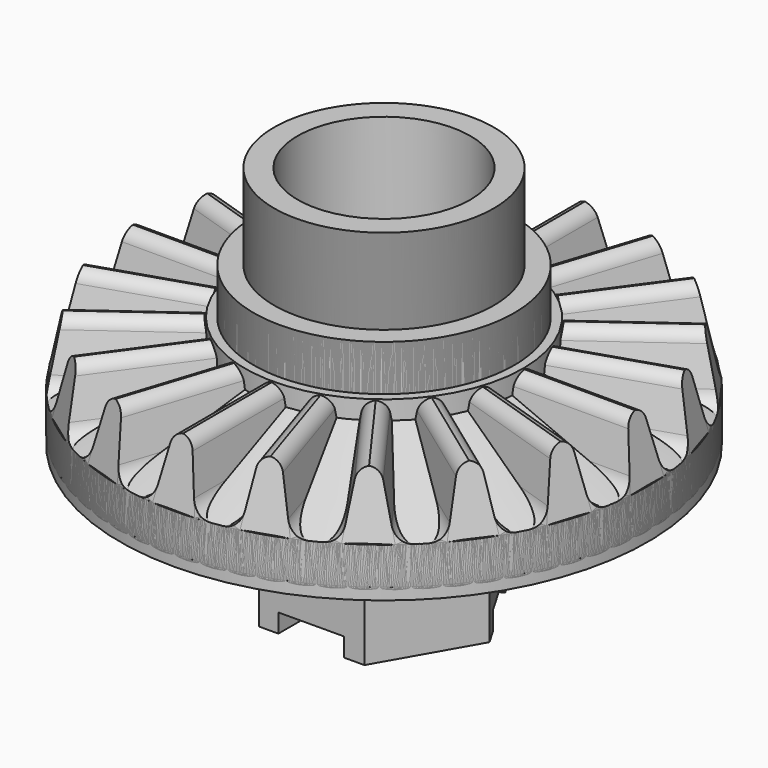
from build123d import *

# Parameters (mm, degrees)
F0_R             = 11.3
F1_DEPTH         = 2.1
F2_R             = 5.575
F3_DEPTH         = 4.67
F4_R             = 4.7
F5_DEPTH         = 3.66
F6_W             = 1.8
F6_H             = 5.7622275918
F7_DEPTH         = 2.7
F7_TAPER         = 10.8
F8_COUNT         = 20
F9_R             = 5.9562746784
F10_DEPTH        = 2.7
F11_T4_DEPTH     = 7.2139383377
F11_T9_DEPTH     = 7.2139383377
F11_2_T4_DEPTH   = 7.2139383377
F11_2_T9_DEPTH   = 7.2139383377
F11_3_T4_DEPTH   = 7.2139383377
F11_3_T9_DEPTH   = 7.2139383377
F11_4_T4_DEPTH   = 7.2139383377
F11_4_T9_DEPTH   = 7.2139383377
F11_5_T4_DEPTH   = 7.2139383377
F11_5_T9_DEPTH   = 7.2139383377
F11_6_T4_DEPTH   = 7.2139383377
F11_6_T9_DEPTH   = 7.2139383377
F11_7_T4_DEPTH   = 7.2139383377
F11_7_T9_DEPTH   = 7.2139383377
F11_8_T4_DEPTH   = 7.2139383377
F11_8_T9_DEPTH   = 7.2139383377
F11_9_T4_DEPTH   = 7.2139383377
F11_9_T9_DEPTH   = 7.2139383377
F11_10_T4_DEPTH  = 7.2139383377
F11_10_T9_DEPTH  = 7.2139383377
F11_11_T4_DEPTH  = 7.2139383377
F11_11_T9_DEPTH  = 7.2139383377
F11_12_T4_DEPTH  = 7.2139383377
F11_12_T9_DEPTH  = 7.2139383377
F11_13_T4_DEPTH  = 7.2139383377
F11_13_T9_DEPTH  = 7.2139383377
F11_14_T4_DEPTH  = 7.2139383377
F11_14_T9_DEPTH  = 7.2139383377
F11_15_T4_DEPTH  = 7.2139383377
F11_15_T9_DEPTH  = 7.2139383377
F11_16_T4_DEPTH  = 7.2139383377
F11_16_T9_DEPTH  = 7.2139383377
F11_17_T4_DEPTH  = 7.2139383377
F11_17_T9_DEPTH  = 7.2139383377
F11_18_T4_DEPTH  = 7.2139383377
F11_18_T9_DEPTH  = 7.2139383377
F11_19_T4_DEPTH  = 7.2139383377
F11_19_T9_DEPTH  = 7.2139383377
F11_20_T4_DEPTH  = 7.2139383377
F11_20_T9_DEPTH  = 7.2139383377
F12_T4_DEPTH     = 9.0713153756
F12_S5_R         = 5.575
F12_T6_DEPTH     = 6
F12_T10_DEPTH    = 9.0713153756
F12_S11_R        = 11.3
F12_T12_DEPTH    = 6
F12_T18_DEPTH    = 9.0713153756
F12_S19_R        = 11.3
F12_T20_DEPTH    = 6
F12_T26_DEPTH    = 9.0713153756
F12_S27_R        = 5.575
F12_T28_DEPTH    = 6
F12_2_T4_DEPTH   = 9.0713153756
F12_2_S5_R       = 5.575
F12_2_T6_DEPTH   = 6
F12_2_T10_DEPTH  = 9.0713153756
F12_2_S11_R      = 11.3
F12_2_T12_DEPTH  = 6
F12_2_T18_DEPTH  = 9.0713153756
F12_2_S19_R      = 11.3
F12_2_T20_DEPTH  = 6
F12_2_T26_DEPTH  = 9.0713153756
F12_2_S27_R      = 5.575
F12_2_T28_DEPTH  = 6
F12_3_T4_DEPTH   = 9.0713153756
F12_3_S5_R       = 5.575
F12_3_T6_DEPTH   = 6
F12_3_T10_DEPTH  = 9.0713153756
F12_3_S11_R      = 11.3
F12_3_T12_DEPTH  = 6
F12_3_T18_DEPTH  = 9.0713153756
F12_3_S19_R      = 11.3
F12_3_T20_DEPTH  = 6
F12_3_T26_DEPTH  = 9.0713153756
F12_3_S27_R      = 5.575
F12_3_T28_DEPTH  = 6
F12_4_T4_DEPTH   = 9.0713153756
F12_4_S5_R       = 5.575
F12_4_T6_DEPTH   = 6
F12_4_T10_DEPTH  = 9.0713153756
F12_4_S11_R      = 11.3
F12_4_T12_DEPTH  = 6
F12_4_T18_DEPTH  = 9.0713153756
F12_4_S19_R      = 11.3
F12_4_T20_DEPTH  = 6
F12_4_T26_DEPTH  = 9.0713153756
F12_4_S27_R      = 5.575
F12_4_T28_DEPTH  = 6
F12_5_T4_DEPTH   = 9.0713153756
F12_5_S5_R       = 5.575
F12_5_T6_DEPTH   = 6
F12_5_T10_DEPTH  = 9.0713153756
F12_5_S11_R      = 11.3
F12_5_T12_DEPTH  = 6
F12_5_T18_DEPTH  = 9.0713153756
F12_5_S19_R      = 11.3
F12_5_T20_DEPTH  = 6
F12_5_T26_DEPTH  = 9.0713153756
F12_5_S27_R      = 5.575
F12_5_T28_DEPTH  = 6
F12_6_T4_DEPTH   = 9.0713153756
F12_6_S5_R       = 5.575
F12_6_T6_DEPTH   = 6
F12_6_T10_DEPTH  = 9.0713153756
F12_6_S11_R      = 11.3
F12_6_T12_DEPTH  = 6
F12_6_T18_DEPTH  = 9.0713153756
F12_6_S19_R      = 11.3
F12_6_T20_DEPTH  = 6
F12_6_T26_DEPTH  = 9.0713153756
F12_6_S27_R      = 5.575
F12_6_T28_DEPTH  = 6
F12_7_T4_DEPTH   = 9.0713153756
F12_7_S5_R       = 5.575
F12_7_T6_DEPTH   = 6
F12_7_T10_DEPTH  = 9.0713153756
F12_7_S11_R      = 11.3
F12_7_T12_DEPTH  = 6
F12_7_T18_DEPTH  = 9.0713153756
F12_7_S19_R      = 11.3
F12_7_T20_DEPTH  = 6
F12_7_T26_DEPTH  = 9.0713153756
F12_7_S27_R      = 5.575
F12_7_T28_DEPTH  = 6
F12_8_T4_DEPTH   = 9.0713153756
F12_8_S5_R       = 5.575
F12_8_T6_DEPTH   = 6
F12_8_T10_DEPTH  = 9.0713153756
F12_8_S11_R      = 11.3
F12_8_T12_DEPTH  = 6
F12_8_T18_DEPTH  = 9.0713153756
F12_8_S19_R      = 11.3
F12_8_T20_DEPTH  = 6
F12_8_T26_DEPTH  = 9.0713153756
F12_8_S27_R      = 5.575
F12_8_T28_DEPTH  = 6
F12_9_T4_DEPTH   = 9.0713153756
F12_9_S5_R       = 5.575
F12_9_T6_DEPTH   = 6
F12_9_T10_DEPTH  = 9.0713153756
F12_9_S11_R      = 11.3
F12_9_T12_DEPTH  = 6
F12_9_T18_DEPTH  = 9.0713153756
F12_9_S19_R      = 11.3
F12_9_T20_DEPTH  = 6
F12_9_T26_DEPTH  = 9.0713153756
F12_9_S27_R      = 5.575
F12_9_T28_DEPTH  = 6
F12_10_T4_DEPTH  = 9.0713153756
F12_10_S5_R      = 5.575
F12_10_T6_DEPTH  = 6
F12_10_T10_DEPTH = 9.0713153756
F12_10_S11_R     = 11.3
F12_10_T12_DEPTH = 6
F12_10_T18_DEPTH = 9.0713153756
F12_10_S19_R     = 11.3
F12_10_T20_DEPTH = 6
F12_10_T26_DEPTH = 9.0713153756
F12_10_S27_R     = 5.575
F12_10_T28_DEPTH = 6
F12_11_T4_DEPTH  = 9.0713153756
F12_11_S5_R      = 11.3
F12_11_T6_DEPTH  = 6
F12_11_T12_DEPTH = 9.0713153756
F12_11_S13_R     = 5.575
F12_11_T14_DEPTH = 6
F12_11_T18_DEPTH = 9.0713153756
F12_11_S19_R     = 5.575
F12_11_T20_DEPTH = 6
F12_11_T24_DEPTH = 9.0713153756
F12_11_S25_R     = 11.3
F12_11_T26_DEPTH = 6
F12_12_T4_DEPTH  = 9.0713153756
F12_12_S5_R      = 11.3
F12_12_T6_DEPTH  = 6
F12_12_T12_DEPTH = 9.0713153756
F12_12_S13_R     = 5.575
F12_12_T14_DEPTH = 6
F12_12_T18_DEPTH = 9.0713153756
F12_12_S19_R     = 5.575
F12_12_T20_DEPTH = 6
F12_12_T24_DEPTH = 9.0713153756
F12_12_S25_R     = 11.3
F12_12_T26_DEPTH = 6
F12_13_T4_DEPTH  = 9.0713153756
F12_13_S5_R      = 11.3
F12_13_T6_DEPTH  = 6
F12_13_T12_DEPTH = 9.0713153756
F12_13_S13_R     = 5.575
F12_13_T14_DEPTH = 6
F12_13_T18_DEPTH = 9.0713153756
F12_13_S19_R     = 5.575
F12_13_T20_DEPTH = 6
F12_13_T24_DEPTH = 9.0713153756
F12_13_S25_R     = 11.3
F12_13_T26_DEPTH = 6
F12_14_T4_DEPTH  = 9.0713153756
F12_14_S5_R      = 11.3
F12_14_T6_DEPTH  = 6
F12_14_T12_DEPTH = 9.0713153756
F12_14_S13_R     = 5.575
F12_14_T14_DEPTH = 6
F12_14_T18_DEPTH = 9.0713153756
F12_14_S19_R     = 5.575
F12_14_T20_DEPTH = 6
F12_14_T24_DEPTH = 9.0713153756
F12_14_S25_R     = 11.3
F12_14_T26_DEPTH = 6
F12_15_T4_DEPTH  = 9.0713153756
F12_15_S5_R      = 11.3
F12_15_T6_DEPTH  = 6
F12_15_T12_DEPTH = 9.0713153756
F12_15_S13_R     = 5.575
F12_15_T14_DEPTH = 6
F12_15_T18_DEPTH = 9.0713153756
F12_15_S19_R     = 5.575
F12_15_T20_DEPTH = 6
F12_15_T24_DEPTH = 9.0713153756
F12_15_S25_R     = 11.3
F12_15_T26_DEPTH = 6
F12_16_T4_DEPTH  = 9.0713153756
F12_16_S5_R      = 11.3
F12_16_T6_DEPTH  = 6
F12_16_T12_DEPTH = 9.0713153756
F12_16_S13_R     = 5.575
F12_16_T14_DEPTH = 6
F12_16_T18_DEPTH = 9.0713153756
F12_16_S19_R     = 5.575
F12_16_T20_DEPTH = 6
F12_16_T24_DEPTH = 9.0713153756
F12_16_S25_R     = 11.3
F12_16_T26_DEPTH = 6
F12_17_T4_DEPTH  = 9.0713153756
F12_17_S5_R      = 11.3
F12_17_T6_DEPTH  = 6
F12_17_T12_DEPTH = 9.0713153756
F12_17_S13_R     = 5.575
F12_17_T14_DEPTH = 6
F12_17_T18_DEPTH = 9.0713153756
F12_17_S19_R     = 5.575
F12_17_T20_DEPTH = 6
F12_17_T24_DEPTH = 9.0713153756
F12_17_S25_R     = 11.3
F12_17_T26_DEPTH = 6
F12_18_T4_DEPTH  = 9.0713153756
F12_18_S5_R      = 11.3
F12_18_T6_DEPTH  = 6
F12_18_T12_DEPTH = 9.0713153756
F12_18_S13_R     = 5.575
F12_18_T14_DEPTH = 6
F12_18_T18_DEPTH = 9.0713153756
F12_18_S19_R     = 5.575
F12_18_T20_DEPTH = 6
F12_18_T24_DEPTH = 9.0713153756
F12_18_S25_R     = 11.3
F12_18_T26_DEPTH = 6
F12_19_T4_DEPTH  = 9.0713153756
F12_19_S5_R      = 5.575
F12_19_T6_DEPTH  = 6
F12_19_T10_DEPTH = 9.0713153756
F12_19_S11_R     = 11.3
F12_19_T12_DEPTH = 6
F12_19_T18_DEPTH = 9.0713153756
F12_19_S19_R     = 11.3
F12_19_T20_DEPTH = 6
F12_19_T26_DEPTH = 9.0713153756
F12_19_S27_R     = 5.575
F12_19_T28_DEPTH = 6
F12_20_T4_DEPTH  = 9.0713153756
F12_20_S5_R      = 5.575
F12_20_T6_DEPTH  = 6
F12_20_T10_DEPTH = 9.0713153756
F12_20_S11_R     = 11.3
F12_20_T12_DEPTH = 6
F12_20_T18_DEPTH = 9.0713153756
F12_20_S19_R     = 11.3
F12_20_T20_DEPTH = 6
F12_20_T26_DEPTH = 9.0713153756
F12_20_S27_R     = 5.575
F12_20_T28_DEPTH = 6
F13_R            = 11.3
F13_R_2          = 5.9562746784
F14_DEPTH        = 2.03
F17_DEPTH        = 6
F18_R            = 2.075
F19_DEPTH        = 25
F20_R            = 3.7
F21_DEPTH        = 10.15
F22_R            = 0.5
F22_2_R          = 0.5
F22_3_R          = 0.5
F22_4_R          = 0.5
F22_5_R          = 0.5
F22_6_R          = 0.5
F22_7_R          = 0.5
F22_8_R          = 0.5
F22_9_R          = 0.5
F22_10_R         = 0.5
F22_11_R         = 0.5
F22_12_R         = 0.5
F22_13_R         = 0.5
F22_14_R         = 0.5
F22_15_R         = 0.5
F22_16_R         = 0.5
F22_17_R         = 0.5
F22_18_R         = 0.5
F22_19_R         = 0.5
F24_DEPTH        = 0.8


# Not quite as in the source:
# - a fillet or chamfer that OpenCascade refuses, or shapes differently, is made with other operations: its cross-section is extruded or revolved along the edge and cut away or added


with BuildPart() as f1:
    # F0 (on Top) → F1 (new body)
    with BuildSketch(Plane.XY):
        Circle(F0_R)
    extrude(amount=F1_DEPTH)

    # F2 (on face) → F3 (join)
    with BuildSketch(Plane.XY.offset(2.1)):
        Circle(F2_R)
    extrude(amount=F3_DEPTH)

    # F4 (on face) → F5 (join)
    with BuildSketch(Plane.XY.offset(6.77)):
        Circle(F4_R)
    extrude(amount=F5_DEPTH)

    # F6 (on face) → F7 (join)
    with BuildSketch(Plane.XY.offset(2.1)):
        with Locations((0, 8.3829884764)):
            Rectangle(F6_W, F6_H)
    extrude(amount=F7_DEPTH, taper=F7_TAPER)


with BuildPart() as f8_1:
    # F8: instance of F1
    add(f1.part.rotate(Axis((0, 0, 2.1), (0, 0, -1)), 1 * 360 / F8_COUNT))

    # F11#2: fillet of radius 0.6 on 2 edges, made by hand


with BuildPart() as f8_2:
    # F8: instance of F1
    add(f1.part.rotate(Axis((0, 0, 2.1), (0, 0, -1)), 2 * 360 / F8_COUNT))

    # F11#3: fillet of radius 0.6 on 2 edges, made by hand


with BuildPart() as f8_3:
    # F8: instance of F1
    add(f1.part.rotate(Axis((0, 0, 2.1), (0, 0, -1)), 3 * 360 / F8_COUNT))

    # F11#4: fillet of radius 0.6 on 2 edges, made by hand


with BuildPart() as f8_4:
    # F8: instance of F1
    add(f1.part.rotate(Axis((0, 0, 2.1), (0, 0, -1)), 4 * 360 / F8_COUNT))

    # F11#5: fillet of radius 0.6 on 2 edges, made by hand


with BuildPart() as f8_5:
    # F8: instance of F1
    add(f1.part.rotate(Axis((0, 0, 2.1), (0, 0, -1)), 5 * 360 / F8_COUNT))

    # F11#6: fillet of radius 0.6 on 2 edges, made by hand


with BuildPart() as f8_6:
    # F8: instance of F1
    add(f1.part.rotate(Axis((0, 0, 2.1), (0, 0, -1)), 6 * 360 / F8_COUNT))

    # F11#7: fillet of radius 0.6 on 2 edges, made by hand


with BuildPart() as f8_7:
    # F8: instance of F1
    add(f1.part.rotate(Axis((0, 0, 2.1), (0, 0, -1)), 7 * 360 / F8_COUNT))

    # F11#8: fillet of radius 0.6 on 2 edges, made by hand


with BuildPart() as f8_8:
    # F8: instance of F1
    add(f1.part.rotate(Axis((0, 0, 2.1), (0, 0, -1)), 8 * 360 / F8_COUNT))

    # F11#9: fillet of radius 0.6 on 2 edges, made by hand


with BuildPart() as f8_9:
    # F8: instance of F1
    add(f1.part.rotate(Axis((0, 0, 2.1), (0, 0, -1)), 9 * 360 / F8_COUNT))

    # F11#10: fillet of radius 0.6 on 2 edges, made by hand


with BuildPart() as f8_10:
    # F8: instance of F1
    add(f1.part.rotate(Axis((0, 0, 2.1), (0, 0, -1)), 10 * 360 / F8_COUNT))

    # F11#11: fillet of radius 0.6 on 2 edges, made by hand


with BuildPart() as f8_11:
    # F8: instance of F1
    add(f1.part.rotate(Axis((0, 0, 2.1), (0, 0, -1)), 11 * 360 / F8_COUNT))

    # F11#12: fillet of radius 0.6 on 2 edges, made by hand


with BuildPart() as f8_12:
    # F8: instance of F1
    add(f1.part.rotate(Axis((0, 0, 2.1), (0, 0, -1)), 12 * 360 / F8_COUNT))

    # F11#13: fillet of radius 0.6 on 2 edges, made by hand


with BuildPart() as f8_13:
    # F8: instance of F1
    add(f1.part.rotate(Axis((0, 0, 2.1), (0, 0, -1)), 13 * 360 / F8_COUNT))

    # F11#14: fillet of radius 0.6 on 2 edges, made by hand


with BuildPart() as f8_14:
    # F8: instance of F1
    add(f1.part.rotate(Axis((0, 0, 2.1), (0, 0, -1)), 14 * 360 / F8_COUNT))

    # F11#15: fillet of radius 0.6 on 2 edges, made by hand


with BuildPart() as f8_15:
    # F8: instance of F1
    add(f1.part.rotate(Axis((0, 0, 2.1), (0, 0, -1)), 15 * 360 / F8_COUNT))

    # F11#16: fillet of radius 0.6 on 2 edges, made by hand


with BuildPart() as f8_16:
    # F8: instance of F1
    add(f1.part.rotate(Axis((0, 0, 2.1), (0, 0, -1)), 16 * 360 / F8_COUNT))

    # F11#17: fillet of radius 0.6 on 2 edges, made by hand


with BuildPart() as f8_17:
    # F8: instance of F1
    add(f1.part.rotate(Axis((0, 0, 2.1), (0, 0, -1)), 17 * 360 / F8_COUNT))

    # F11#18: fillet of radius 0.6 on 2 edges, made by hand


with BuildPart() as f8_18:
    # F8: instance of F1
    add(f1.part.rotate(Axis((0, 0, 2.1), (0, 0, -1)), 18 * 360 / F8_COUNT))

    # F11#19: fillet of radius 0.6 on 2 edges, made by hand


with BuildPart() as f8_19:
    # F8: instance of F1
    add(f1.part.rotate(Axis((0, 0, 2.1), (0, 0, -1)), 19 * 360 / F8_COUNT))

    # F11#20: fillet of radius 0.6 on 2 edges, made by hand


with BuildPart() as f10:
    # F9 (on face) → F10 (new body)
    with BuildSketch(Plane.XY.offset(2.1)):
        Circle(F9_R)
    extrude(amount=F10_DEPTH)


with BuildPart() as f1_1:
    add(f1.part)

    # F11: fillet of radius 0.6 on 2 edges, made by hand


with BuildPart() as f11_tool2:
    # F11_s3 → F11_t4 (new body)
    with BuildSketch(Plane.XZ.offset(-4.7760193075)):
        with BuildLine():
            ThreePointArc((0.4779566369, 4.3124287888), (0.2710386803, 4.6623079457), (-0.1114157136, 4.8))
            Line((-0.1114157136, 4.8), (0.384947454, 4.8))
            Line((0.384947454, 4.8), (0.4779566369, 4.3124287888))
        make_face()
    extrude(amount=-F11_T4_DEPTH)

    split(bisect_by=Plane(origin=(0, 4.9221634131, -0.938952888), x_dir=(1, 0, 0), z_dir=(0, 0.9822872507, -0.1873813146)), keep=Keep.TOP)


with BuildPart() as f1_2:
    add(f1_1.part)

    # F11_t1: cut F11_tool2
    add(f11_tool2.part, mode=Mode.SUBTRACT)


with BuildPart() as f11_tool7:
    # F11_s8 → F11_t9 (new body)
    with BuildSketch(Plane.XZ.offset(-11.9899576452)):
        with BuildLine():
            ThreePointArc((-0.4779566369, 4.3124287888), (-0.2710386803, 4.6623079457), (0.1114157136, 4.8))
            Line((0.1114157136, 4.8), (-0.384947454, 4.8))
            Line((-0.384947454, 4.8), (-0.4779566369, 4.3124287888))
        make_face()
    extrude(amount=F11_T9_DEPTH)

    split(bisect_by=Plane(origin=(0, 4.9221634131, -0.938952888), x_dir=(1, 0, 0), z_dir=(0, 0.9822872507, -0.1873813146)), keep=Keep.TOP)


with BuildPart() as f1_3:
    add(f1_2.part)

    # F11_t6: cut F11_tool7
    add(f11_tool7.part, mode=Mode.SUBTRACT)

    # F12: fillet of radius 0.8 on 2 edges, made by hand


with BuildPart() as f11_2_tool2:
    # F11_2_s3 → F11_2_t4 (new body)
    with BuildSketch(Plane(origin=(3.7051006742, 11.4031273486, 0), x_dir=(0, 0, 1), z_dir=(-0.3090169944, -0.9510565163, 0))):
        with BuildLine():
            ThreePointArc((4.3124287888, 0.4779566369), (4.6623079457, 0.2710386803), (4.8, -0.1114157136))
            Line((4.8, -0.1114157136), (4.8, 0.384947454))
            Line((4.8, 0.384947454), (4.3124287888, 0.4779566369))
        make_face()
    extrude(amount=F11_2_T4_DEPTH)

    split(bisect_by=Plane(origin=(1.5210321437, 4.6812555883, -0.938952888), x_dir=(-0.9510565163, 0.3090169944, 0), z_dir=(0.3035434538, 0.9342106907, -0.1873813146)), keep=Keep.TOP)


with BuildPart() as f8_1_1:
    add(f8_1.part)

    # F11_2_t1: cut F11_2_tool2
    add(f11_2_tool2.part, mode=Mode.SUBTRACT)


with BuildPart() as f11_2_tool7:
    # F11_2_s8 → F11_2_t9 (new body)
    with BuildSketch(Plane(origin=(1.4758711315, 4.5422642844, 0), x_dir=(0, 0, 1), z_dir=(0.3090169944, 0.9510565163, 0))):
        with BuildLine():
            ThreePointArc((4.3124287888, 0.4779566369), (4.6623079457, 0.2710386803), (4.8, -0.1114157136))
            Line((4.8, -0.1114157136), (4.8, 0.384947454))
            Line((4.8, 0.384947454), (4.3124287888, 0.4779566369))
        make_face()
    extrude(amount=F11_2_T9_DEPTH)

    split(bisect_by=Plane(origin=(1.5210321437, 4.6812555883, -0.938952888), x_dir=(-0.9510565163, 0.3090169944, 0), z_dir=(0.3035434538, 0.9342106907, -0.1873813146)), keep=Keep.TOP)


with BuildPart() as f8_1_2:
    add(f8_1_1.part)

    # F11_2_t6: cut F11_2_tool7
    add(f11_2_tool7.part, mode=Mode.SUBTRACT)

    # F12#2: fillet of radius 0.8 on 2 edges, made by hand


with BuildPart() as f11_3_tool2:
    # F11_3_s3 → F11_3_t4 (new body)
    with BuildSketch(Plane(origin=(7.0475202795, 9.7000794968, 0), x_dir=(0, 0, 1), z_dir=(-0.5877852523, -0.8090169944, 0))):
        with BuildLine():
            ThreePointArc((4.3124287888, 0.4779566369), (4.6623079457, 0.2710386803), (4.8, -0.1114157136))
            Line((4.8, -0.1114157136), (4.8, 0.384947454))
            Line((4.8, 0.384947454), (4.3124287888, 0.4779566369))
        make_face()
    extrude(amount=F11_3_T4_DEPTH)

    split(bisect_by=Plane(origin=(2.8931750636, 3.9821138503, -0.938952888), x_dir=(-0.8090169944, 0.5877852523, 0), z_dir=(0.5773739595, 0.7946870792, -0.1873813146)), keep=Keep.TOP)


with BuildPart() as f8_2_1:
    add(f8_2.part)

    # F11_3_t1: cut F11_3_tool2
    add(f11_3_tool2.part, mode=Mode.SUBTRACT)


with BuildPart() as f11_3_tool7:
    # F11_3_s8 → F11_3_t9 (new body)
    with BuildSketch(Plane(origin=(2.8072737136, 3.8638807853, 0), x_dir=(0, 0, 1), z_dir=(0.5877852523, 0.8090169944, 0))):
        with BuildLine():
            ThreePointArc((4.3124287888, 0.4779566369), (4.6623079457, 0.2710386803), (4.8, -0.1114157136))
            Line((4.8, -0.1114157136), (4.8, 0.384947454))
            Line((4.8, 0.384947454), (4.3124287888, 0.4779566369))
        make_face()
    extrude(amount=F11_3_T9_DEPTH)

    split(bisect_by=Plane(origin=(2.8931750636, 3.9821138503, -0.938952888), x_dir=(-0.8090169944, 0.5877852523, 0), z_dir=(0.5773739595, 0.7946870792, -0.1873813146)), keep=Keep.TOP)


with BuildPart() as f8_2_2:
    add(f8_2_1.part)

    # F11_3_t6: cut F11_3_tool7
    add(f11_3_tool7.part, mode=Mode.SUBTRACT)

    # F12#3: fillet of radius 0.8 on 2 edges, made by hand


with BuildPart() as f11_4_tool2:
    # F11_4_s3 → F11_4_t4 (new body)
    with BuildSketch(Plane(origin=(9.7000794968, 7.0475202795, 0), x_dir=(0, 0, 1), z_dir=(-0.8090169944, -0.5877852523, 0))):
        with BuildLine():
            ThreePointArc((4.3124287888, 0.4779566369), (4.6623079457, 0.2710386803), (4.8, -0.1114157136))
            Line((4.8, -0.1114157136), (4.8, 0.384947454))
            Line((4.8, 0.384947454), (4.3124287888, 0.4779566369))
        make_face()
    extrude(amount=F11_4_T4_DEPTH)

    split(bisect_by=Plane(origin=(3.9821138503, 2.8931750636, -0.938952888), x_dir=(-0.5877852523, 0.8090169944, 0), z_dir=(0.7946870792, 0.5773739595, -0.1873813146)), keep=Keep.TOP)


with BuildPart() as f8_3_1:
    add(f8_3.part)

    # F11_4_t1: cut F11_4_tool2
    add(f11_4_tool2.part, mode=Mode.SUBTRACT)


with BuildPart() as f11_4_tool7:
    # F11_4_s8 → F11_4_t9 (new body)
    with BuildSketch(Plane(origin=(3.8638807853, 2.8072737136, 0), x_dir=(0, 0, 1), z_dir=(0.8090169944, 0.5877852523, 0))):
        with BuildLine():
            ThreePointArc((4.3124287888, 0.4779566369), (4.6623079457, 0.2710386803), (4.8, -0.1114157136))
            Line((4.8, -0.1114157136), (4.8, 0.384947454))
            Line((4.8, 0.384947454), (4.3124287888, 0.4779566369))
        make_face()
    extrude(amount=F11_4_T9_DEPTH)

    split(bisect_by=Plane(origin=(3.9821138503, 2.8931750636, -0.938952888), x_dir=(-0.5877852523, 0.8090169944, 0), z_dir=(0.7946870792, 0.5773739595, -0.1873813146)), keep=Keep.TOP)


with BuildPart() as f8_3_2:
    add(f8_3_1.part)

    # F11_4_t6: cut F11_4_tool7
    add(f11_4_tool7.part, mode=Mode.SUBTRACT)

    # F12#4: fillet of radius 0.8 on 2 edges, made by hand


with BuildPart() as f11_5_tool2:
    # F11_5_s3 → F11_5_t4 (new body)
    with BuildSketch(Plane(origin=(4.5422642844, 1.4758711315, 0), x_dir=(0, 0, 1), z_dir=(0.9510565163, 0.3090169944, 0))):
        with BuildLine():
            ThreePointArc((4.3124287888, 0.4779566369), (4.6623079457, 0.2710386803), (4.8, -0.1114157136))
            Line((4.8, -0.1114157136), (4.8, 0.384947454))
            Line((4.8, 0.384947454), (4.3124287888, 0.4779566369))
        make_face()
    extrude(amount=F11_5_T4_DEPTH)

    split(bisect_by=Plane(origin=(4.6812555883, 1.5210321437, -0.938952888), x_dir=(-0.3090169944, 0.9510565163, 0), z_dir=(0.9342106907, 0.3035434538, -0.1873813146)), keep=Keep.TOP)


with BuildPart() as f8_4_1:
    add(f8_4.part)

    # F11_5_t1: cut F11_5_tool2
    add(f11_5_tool2.part, mode=Mode.SUBTRACT)


with BuildPart() as f11_5_tool7:
    # F11_5_s8 → F11_5_t9 (new body)
    with BuildSketch(Plane(origin=(11.4031273486, 3.7051006742, 0), x_dir=(0, 0, 1), z_dir=(-0.9510565163, -0.3090169944, 0))):
        with BuildLine():
            ThreePointArc((4.3124287888, 0.4779566369), (4.6623079457, 0.2710386803), (4.8, -0.1114157136))
            Line((4.8, -0.1114157136), (4.8, 0.384947454))
            Line((4.8, 0.384947454), (4.3124287888, 0.4779566369))
        make_face()
    extrude(amount=F11_5_T9_DEPTH)

    split(bisect_by=Plane(origin=(4.6812555883, 1.5210321437, -0.938952888), x_dir=(-0.3090169944, 0.9510565163, 0), z_dir=(0.9342106907, 0.3035434538, -0.1873813146)), keep=Keep.TOP)


with BuildPart() as f8_4_2:
    add(f8_4_1.part)

    # F11_5_t6: cut F11_5_tool7
    add(f11_5_tool7.part, mode=Mode.SUBTRACT)

    # F12#5: fillet of radius 0.8 on 2 edges, made by hand


with BuildPart() as f11_6_tool2:
    # F11_6_s3 → F11_6_t4 (new body)
    with BuildSketch(Plane.YZ.offset(11.9899576452)):
        with BuildLine():
            ThreePointArc((0.4779566369, 4.3124287888), (0.2710386803, 4.6623079457), (-0.1114157136, 4.8))
            Line((-0.1114157136, 4.8), (0.384947454, 4.8))
            Line((0.384947454, 4.8), (0.4779566369, 4.3124287888))
        make_face()
    extrude(amount=-F11_6_T4_DEPTH)

    split(bisect_by=Plane(origin=(4.9221634131, 0, -0.938952888), x_dir=(0, 1, 0), z_dir=(0.9822872507, 0, -0.1873813146)), keep=Keep.TOP)


with BuildPart() as f8_5_1:
    add(f8_5.part)

    # F11_6_t1: cut F11_6_tool2
    add(f11_6_tool2.part, mode=Mode.SUBTRACT)


with BuildPart() as f11_6_tool7:
    # F11_6_s8 → F11_6_t9 (new body)
    with BuildSketch(Plane.YZ.offset(4.7760193075)):
        with BuildLine():
            ThreePointArc((-0.4779566369, 4.3124287888), (-0.2710386803, 4.6623079457), (0.1114157136, 4.8))
            Line((0.1114157136, 4.8), (-0.384947454, 4.8))
            Line((-0.384947454, 4.8), (-0.4779566369, 4.3124287888))
        make_face()
    extrude(amount=F11_6_T9_DEPTH)

    split(bisect_by=Plane(origin=(4.9221634131, 0, -0.938952888), x_dir=(0, 1, 0), z_dir=(0.9822872507, 0, -0.1873813146)), keep=Keep.TOP)


with BuildPart() as f8_5_2:
    add(f8_5_1.part)

    # F11_6_t6: cut F11_6_tool7
    add(f11_6_tool7.part, mode=Mode.SUBTRACT)

    # F12#6: fillet of radius 0.8 on 2 edges, made by hand


with BuildPart() as f11_7_tool2:
    # F11_7_s3 → F11_7_t4 (new body)
    with BuildSketch(Plane(origin=(11.4031273486, -3.7051006742, 0), x_dir=(0, 0, 1), z_dir=(-0.9510565163, 0.3090169944, 0))):
        with BuildLine():
            ThreePointArc((4.3124287888, 0.4779566369), (4.6623079457, 0.2710386803), (4.8, -0.1114157136))
            Line((4.8, -0.1114157136), (4.8, 0.384947454))
            Line((4.8, 0.384947454), (4.3124287888, 0.4779566369))
        make_face()
    extrude(amount=F11_7_T4_DEPTH)

    split(bisect_by=Plane(origin=(4.6812555883, -1.5210321437, -0.938952888), x_dir=(0.3090169944, 0.9510565163, 0), z_dir=(0.9342106907, -0.3035434538, -0.1873813146)), keep=Keep.TOP)


with BuildPart() as f8_6_1:
    add(f8_6.part)

    # F11_7_t1: cut F11_7_tool2
    add(f11_7_tool2.part, mode=Mode.SUBTRACT)


with BuildPart() as f11_7_tool7:
    # F11_7_s8 → F11_7_t9 (new body)
    with BuildSketch(Plane(origin=(4.5422642844, -1.4758711315, 0), x_dir=(0, 0, 1), z_dir=(0.9510565163, -0.3090169944, 0))):
        with BuildLine():
            ThreePointArc((4.3124287888, 0.4779566369), (4.6623079457, 0.2710386803), (4.8, -0.1114157136))
            Line((4.8, -0.1114157136), (4.8, 0.384947454))
            Line((4.8, 0.384947454), (4.3124287888, 0.4779566369))
        make_face()
    extrude(amount=F11_7_T9_DEPTH)

    split(bisect_by=Plane(origin=(4.6812555883, -1.5210321437, -0.938952888), x_dir=(0.3090169944, 0.9510565163, 0), z_dir=(0.9342106907, -0.3035434538, -0.1873813146)), keep=Keep.TOP)


with BuildPart() as f8_6_2:
    add(f8_6_1.part)

    # F11_7_t6: cut F11_7_tool7
    add(f11_7_tool7.part, mode=Mode.SUBTRACT)

    # F12#7: fillet of radius 0.8 on 2 edges, made by hand


with BuildPart() as f11_8_tool2:
    # F11_8_s3 → F11_8_t4 (new body)
    with BuildSketch(Plane(origin=(9.7000794968, -7.0475202795, 0), x_dir=(0, 0, 1), z_dir=(-0.8090169944, 0.5877852523, 0))):
        with BuildLine():
            ThreePointArc((4.3124287888, 0.4779566369), (4.6623079457, 0.2710386803), (4.8, -0.1114157136))
            Line((4.8, -0.1114157136), (4.8, 0.384947454))
            Line((4.8, 0.384947454), (4.3124287888, 0.4779566369))
        make_face()
    extrude(amount=F11_8_T4_DEPTH)

    split(bisect_by=Plane(origin=(3.9821138503, -2.8931750636, -0.938952888), x_dir=(0.5877852523, 0.8090169944, 0), z_dir=(0.7946870792, -0.5773739595, -0.1873813146)), keep=Keep.TOP)


with BuildPart() as f8_7_1:
    add(f8_7.part)

    # F11_8_t1: cut F11_8_tool2
    add(f11_8_tool2.part, mode=Mode.SUBTRACT)


with BuildPart() as f11_8_tool7:
    # F11_8_s8 → F11_8_t9 (new body)
    with BuildSketch(Plane(origin=(3.8638807853, -2.8072737136, 0), x_dir=(0, 0, 1), z_dir=(0.8090169944, -0.5877852523, 0))):
        with BuildLine():
            ThreePointArc((4.3124287888, 0.4779566369), (4.6623079457, 0.2710386803), (4.8, -0.1114157136))
            Line((4.8, -0.1114157136), (4.8, 0.384947454))
            Line((4.8, 0.384947454), (4.3124287888, 0.4779566369))
        make_face()
    extrude(amount=F11_8_T9_DEPTH)

    split(bisect_by=Plane(origin=(3.9821138503, -2.8931750636, -0.938952888), x_dir=(0.5877852523, 0.8090169944, 0), z_dir=(0.7946870792, -0.5773739595, -0.1873813146)), keep=Keep.TOP)


with BuildPart() as f8_7_2:
    add(f8_7_1.part)

    # F11_8_t6: cut F11_8_tool7
    add(f11_8_tool7.part, mode=Mode.SUBTRACT)

    # F12#8: fillet of radius 0.8 on 2 edges, made by hand


with BuildPart() as f11_9_tool2:
    # F11_9_s3 → F11_9_t4 (new body)
    with BuildSketch(Plane(origin=(7.0475202795, -9.7000794968, 0), x_dir=(0, 0, 1), z_dir=(-0.5877852523, 0.8090169944, 0))):
        with BuildLine():
            ThreePointArc((4.3124287888, 0.4779566369), (4.6623079457, 0.2710386803), (4.8, -0.1114157136))
            Line((4.8, -0.1114157136), (4.8, 0.384947454))
            Line((4.8, 0.384947454), (4.3124287888, 0.4779566369))
        make_face()
    extrude(amount=F11_9_T4_DEPTH)

    split(bisect_by=Plane(origin=(2.8931750636, -3.9821138503, -0.938952888), x_dir=(0.8090169944, 0.5877852523, 0), z_dir=(0.5773739595, -0.7946870792, -0.1873813146)), keep=Keep.TOP)


with BuildPart() as f8_8_1:
    add(f8_8.part)

    # F11_9_t1: cut F11_9_tool2
    add(f11_9_tool2.part, mode=Mode.SUBTRACT)


with BuildPart() as f11_9_tool7:
    # F11_9_s8 → F11_9_t9 (new body)
    with BuildSketch(Plane(origin=(2.8072737136, -3.8638807853, 0), x_dir=(0, 0, 1), z_dir=(0.5877852523, -0.8090169944, 0))):
        with BuildLine():
            ThreePointArc((4.3124287888, 0.4779566369), (4.6623079457, 0.2710386803), (4.8, -0.1114157136))
            Line((4.8, -0.1114157136), (4.8, 0.384947454))
            Line((4.8, 0.384947454), (4.3124287888, 0.4779566369))
        make_face()
    extrude(amount=F11_9_T9_DEPTH)

    split(bisect_by=Plane(origin=(2.8931750636, -3.9821138503, -0.938952888), x_dir=(0.8090169944, 0.5877852523, 0), z_dir=(0.5773739595, -0.7946870792, -0.1873813146)), keep=Keep.TOP)


with BuildPart() as f8_8_2:
    add(f8_8_1.part)

    # F11_9_t6: cut F11_9_tool7
    add(f11_9_tool7.part, mode=Mode.SUBTRACT)

    # F12#9: fillet of radius 0.8 on 2 edges, made by hand


with BuildPart() as f11_10_tool2:
    # F11_10_s3 → F11_10_t4 (new body)
    with BuildSketch(Plane(origin=(3.7051006742, -11.4031273486, 0), x_dir=(0, 0, 1), z_dir=(-0.3090169944, 0.9510565163, 0))):
        with BuildLine():
            ThreePointArc((4.3124287888, 0.4779566369), (4.6623079457, 0.2710386803), (4.8, -0.1114157136))
            Line((4.8, -0.1114157136), (4.8, 0.384947454))
            Line((4.8, 0.384947454), (4.3124287888, 0.4779566369))
        make_face()
    extrude(amount=F11_10_T4_DEPTH)

    split(bisect_by=Plane(origin=(1.5210321437, -4.6812555883, -0.938952888), x_dir=(0.9510565163, 0.3090169944, 0), z_dir=(0.3035434538, -0.9342106907, -0.1873813146)), keep=Keep.TOP)


with BuildPart() as f8_9_1:
    add(f8_9.part)

    # F11_10_t1: cut F11_10_tool2
    add(f11_10_tool2.part, mode=Mode.SUBTRACT)


with BuildPart() as f11_10_tool7:
    # F11_10_s8 → F11_10_t9 (new body)
    with BuildSketch(Plane(origin=(1.4758711315, -4.5422642844, 0), x_dir=(0, 0, 1), z_dir=(0.3090169944, -0.9510565163, 0))):
        with BuildLine():
            ThreePointArc((4.3124287888, 0.4779566369), (4.6623079457, 0.2710386803), (4.8, -0.1114157136))
            Line((4.8, -0.1114157136), (4.8, 0.384947454))
            Line((4.8, 0.384947454), (4.3124287888, 0.4779566369))
        make_face()
    extrude(amount=F11_10_T9_DEPTH)

    split(bisect_by=Plane(origin=(1.5210321437, -4.6812555883, -0.938952888), x_dir=(0.9510565163, 0.3090169944, 0), z_dir=(0.3035434538, -0.9342106907, -0.1873813146)), keep=Keep.TOP)


with BuildPart() as f8_9_2:
    add(f8_9_1.part)

    # F11_10_t6: cut F11_10_tool7
    add(f11_10_tool7.part, mode=Mode.SUBTRACT)

    # F12#10: fillet of radius 0.8 on 2 edges, made by hand


with BuildPart() as f11_11_tool2:
    # F11_11_s3 → F11_11_t4 (new body)
    with BuildSketch(Plane.XZ.offset(11.9899576452)):
        with BuildLine():
            ThreePointArc((0.4779566369, 4.3124287888), (0.2710386803, 4.6623079457), (-0.1114157136, 4.8))
            Line((-0.1114157136, 4.8), (0.384947454, 4.8))
            Line((0.384947454, 4.8), (0.4779566369, 4.3124287888))
        make_face()
    extrude(amount=-F11_11_T4_DEPTH)

    split(bisect_by=Plane(origin=(0, -4.9221634131, -0.938952888), x_dir=(1, 0, 0), z_dir=(0, -0.9822872507, -0.1873813146)), keep=Keep.TOP)


with BuildPart() as f8_10_1:
    add(f8_10.part)

    # F11_11_t1: cut F11_11_tool2
    add(f11_11_tool2.part, mode=Mode.SUBTRACT)


with BuildPart() as f11_11_tool7:
    # F11_11_s8 → F11_11_t9 (new body)
    with BuildSketch(Plane.XZ.offset(4.7760193075)):
        with BuildLine():
            ThreePointArc((-0.4779566369, 4.3124287888), (-0.2710386803, 4.6623079457), (0.1114157136, 4.8))
            Line((0.1114157136, 4.8), (-0.384947454, 4.8))
            Line((-0.384947454, 4.8), (-0.4779566369, 4.3124287888))
        make_face()
    extrude(amount=F11_11_T9_DEPTH)

    split(bisect_by=Plane(origin=(0, -4.9221634131, -0.938952888), x_dir=(1, 0, 0), z_dir=(0, -0.9822872507, -0.1873813146)), keep=Keep.TOP)


with BuildPart() as f8_10_2:
    add(f8_10_1.part)

    # F11_11_t6: cut F11_11_tool7
    add(f11_11_tool7.part, mode=Mode.SUBTRACT)

    # F12#11: fillet of radius 0.8 on 2 edges, made by hand


with BuildPart() as f11_12_tool2:
    # F11_12_s3 → F11_12_t4 (new body)
    with BuildSketch(Plane(origin=(-3.7051006742, -11.4031273486, 0), x_dir=(0, 0, 1), z_dir=(0.3090169944, 0.9510565163, 0))):
        with BuildLine():
            ThreePointArc((4.3124287888, 0.4779566369), (4.6623079457, 0.2710386803), (4.8, -0.1114157136))
            Line((4.8, -0.1114157136), (4.8, 0.384947454))
            Line((4.8, 0.384947454), (4.3124287888, 0.4779566369))
        make_face()
    extrude(amount=F11_12_T4_DEPTH)

    split(bisect_by=Plane(origin=(-1.5210321437, -4.6812555883, -0.938952888), x_dir=(0.9510565163, -0.3090169944, 0), z_dir=(-0.3035434538, -0.9342106907, -0.1873813146)), keep=Keep.TOP)


with BuildPart() as f8_11_1:
    add(f8_11.part)

    # F11_12_t1: cut F11_12_tool2
    add(f11_12_tool2.part, mode=Mode.SUBTRACT)


with BuildPart() as f11_12_tool7:
    # F11_12_s8 → F11_12_t9 (new body)
    with BuildSketch(Plane(origin=(-1.4758711315, -4.5422642844, 0), x_dir=(0, 0, 1), z_dir=(-0.3090169944, -0.9510565163, 0))):
        with BuildLine():
            ThreePointArc((4.3124287888, 0.4779566369), (4.6623079457, 0.2710386803), (4.8, -0.1114157136))
            Line((4.8, -0.1114157136), (4.8, 0.384947454))
            Line((4.8, 0.384947454), (4.3124287888, 0.4779566369))
        make_face()
    extrude(amount=F11_12_T9_DEPTH)

    split(bisect_by=Plane(origin=(-1.5210321437, -4.6812555883, -0.938952888), x_dir=(0.9510565163, -0.3090169944, 0), z_dir=(-0.3035434538, -0.9342106907, -0.1873813146)), keep=Keep.TOP)


with BuildPart() as f8_11_2:
    add(f8_11_1.part)

    # F11_12_t6: cut F11_12_tool7
    add(f11_12_tool7.part, mode=Mode.SUBTRACT)

    # F12#12: fillet of radius 0.8 on 2 edges, made by hand


with BuildPart() as f11_13_tool2:
    # F11_13_s3 → F11_13_t4 (new body)
    with BuildSketch(Plane(origin=(-7.0475202795, -9.7000794968, 0), x_dir=(0, 0, 1), z_dir=(0.5877852523, 0.8090169944, 0))):
        with BuildLine():
            ThreePointArc((4.3124287888, 0.4779566369), (4.6623079457, 0.2710386803), (4.8, -0.1114157136))
            Line((4.8, -0.1114157136), (4.8, 0.384947454))
            Line((4.8, 0.384947454), (4.3124287888, 0.4779566369))
        make_face()
    extrude(amount=F11_13_T4_DEPTH)

    split(bisect_by=Plane(origin=(-2.8931750636, -3.9821138503, -0.938952888), x_dir=(0.8090169944, -0.5877852523, 0), z_dir=(-0.5773739595, -0.7946870792, -0.1873813146)), keep=Keep.TOP)


with BuildPart() as f8_12_1:
    add(f8_12.part)

    # F11_13_t1: cut F11_13_tool2
    add(f11_13_tool2.part, mode=Mode.SUBTRACT)


with BuildPart() as f11_13_tool7:
    # F11_13_s8 → F11_13_t9 (new body)
    with BuildSketch(Plane(origin=(-2.8072737136, -3.8638807853, 0), x_dir=(0, 0, 1), z_dir=(-0.5877852523, -0.8090169944, 0))):
        with BuildLine():
            ThreePointArc((4.3124287888, 0.4779566369), (4.6623079457, 0.2710386803), (4.8, -0.1114157136))
            Line((4.8, -0.1114157136), (4.8, 0.384947454))
            Line((4.8, 0.384947454), (4.3124287888, 0.4779566369))
        make_face()
    extrude(amount=F11_13_T9_DEPTH)

    split(bisect_by=Plane(origin=(-2.8931750636, -3.9821138503, -0.938952888), x_dir=(0.8090169944, -0.5877852523, 0), z_dir=(-0.5773739595, -0.7946870792, -0.1873813146)), keep=Keep.TOP)


with BuildPart() as f8_12_2:
    add(f8_12_1.part)

    # F11_13_t6: cut F11_13_tool7
    add(f11_13_tool7.part, mode=Mode.SUBTRACT)

    # F12#13: fillet of radius 0.8 on 2 edges, made by hand


with BuildPart() as f11_14_tool2:
    # F11_14_s3 → F11_14_t4 (new body)
    with BuildSketch(Plane(origin=(-9.7000794968, -7.0475202795, 0), x_dir=(0, 0, 1), z_dir=(0.8090169944, 0.5877852523, 0))):
        with BuildLine():
            ThreePointArc((4.3124287888, 0.4779566369), (4.6623079457, 0.2710386803), (4.8, -0.1114157136))
            Line((4.8, -0.1114157136), (4.8, 0.384947454))
            Line((4.8, 0.384947454), (4.3124287888, 0.4779566369))
        make_face()
    extrude(amount=F11_14_T4_DEPTH)

    split(bisect_by=Plane(origin=(-3.9821138503, -2.8931750636, -0.938952888), x_dir=(0.5877852523, -0.8090169944, 0), z_dir=(-0.7946870792, -0.5773739595, -0.1873813146)), keep=Keep.TOP)


with BuildPart() as f8_13_1:
    add(f8_13.part)

    # F11_14_t1: cut F11_14_tool2
    add(f11_14_tool2.part, mode=Mode.SUBTRACT)


with BuildPart() as f11_14_tool7:
    # F11_14_s8 → F11_14_t9 (new body)
    with BuildSketch(Plane(origin=(-3.8638807853, -2.8072737136, 0), x_dir=(0, 0, 1), z_dir=(-0.8090169944, -0.5877852523, 0))):
        with BuildLine():
            ThreePointArc((4.3124287888, 0.4779566369), (4.6623079457, 0.2710386803), (4.8, -0.1114157136))
            Line((4.8, -0.1114157136), (4.8, 0.384947454))
            Line((4.8, 0.384947454), (4.3124287888, 0.4779566369))
        make_face()
    extrude(amount=F11_14_T9_DEPTH)

    split(bisect_by=Plane(origin=(-3.9821138503, -2.8931750636, -0.938952888), x_dir=(0.5877852523, -0.8090169944, 0), z_dir=(-0.7946870792, -0.5773739595, -0.1873813146)), keep=Keep.TOP)


with BuildPart() as f8_13_2:
    add(f8_13_1.part)

    # F11_14_t6: cut F11_14_tool7
    add(f11_14_tool7.part, mode=Mode.SUBTRACT)

    # F12#14: fillet of radius 0.8 on 2 edges, made by hand


with BuildPart() as f11_15_tool2:
    # F11_15_s3 → F11_15_t4 (new body)
    with BuildSketch(Plane(origin=(-11.4031273486, -3.7051006742, 0), x_dir=(0, 0, 1), z_dir=(0.9510565163, 0.3090169944, 0))):
        with BuildLine():
            ThreePointArc((4.3124287888, 0.4779566369), (4.6623079457, 0.2710386803), (4.8, -0.1114157136))
            Line((4.8, -0.1114157136), (4.8, 0.384947454))
            Line((4.8, 0.384947454), (4.3124287888, 0.4779566369))
        make_face()
    extrude(amount=F11_15_T4_DEPTH)

    split(bisect_by=Plane(origin=(-4.6812555883, -1.5210321437, -0.938952888), x_dir=(0.3090169944, -0.9510565163, 0), z_dir=(-0.9342106907, -0.3035434538, -0.1873813146)), keep=Keep.TOP)


with BuildPart() as f8_14_1:
    add(f8_14.part)

    # F11_15_t1: cut F11_15_tool2
    add(f11_15_tool2.part, mode=Mode.SUBTRACT)


with BuildPart() as f11_15_tool7:
    # F11_15_s8 → F11_15_t9 (new body)
    with BuildSketch(Plane(origin=(-4.5422642844, -1.4758711315, 0), x_dir=(0, 0, 1), z_dir=(-0.9510565163, -0.3090169944, 0))):
        with BuildLine():
            ThreePointArc((4.3124287888, 0.4779566369), (4.6623079457, 0.2710386803), (4.8, -0.1114157136))
            Line((4.8, -0.1114157136), (4.8, 0.384947454))
            Line((4.8, 0.384947454), (4.3124287888, 0.4779566369))
        make_face()
    extrude(amount=F11_15_T9_DEPTH)

    split(bisect_by=Plane(origin=(-4.6812555883, -1.5210321437, -0.938952888), x_dir=(0.3090169944, -0.9510565163, 0), z_dir=(-0.9342106907, -0.3035434538, -0.1873813146)), keep=Keep.TOP)


with BuildPart() as f8_14_2:
    add(f8_14_1.part)

    # F11_15_t6: cut F11_15_tool7
    add(f11_15_tool7.part, mode=Mode.SUBTRACT)

    # F12#15: fillet of radius 0.8 on 2 edges, made by hand


with BuildPart() as f11_16_tool2:
    # F11_16_s3 → F11_16_t4 (new body)
    with BuildSketch(Plane.YZ.offset(-11.9899576452)):
        with BuildLine():
            ThreePointArc((-0.4779566369, 4.3124287888), (-0.2710386803, 4.6623079457), (0.1114157136, 4.8))
            Line((0.1114157136, 4.8), (-0.384947454, 4.8))
            Line((-0.384947454, 4.8), (-0.4779566369, 4.3124287888))
        make_face()
    extrude(amount=F11_16_T4_DEPTH)

    split(bisect_by=Plane(origin=(-4.9221634131, 0, -0.938952888), x_dir=(0, 1, 0), z_dir=(-0.9822872507, 0, -0.1873813146)), keep=Keep.TOP)


with BuildPart() as f8_15_1:
    add(f8_15.part)

    # F11_16_t1: cut F11_16_tool2
    add(f11_16_tool2.part, mode=Mode.SUBTRACT)


with BuildPart() as f11_16_tool7:
    # F11_16_s8 → F11_16_t9 (new body)
    with BuildSketch(Plane.YZ.offset(-4.7760193075)):
        with BuildLine():
            ThreePointArc((0.4779566369, 4.3124287888), (0.2710386803, 4.6623079457), (-0.1114157136, 4.8))
            Line((-0.1114157136, 4.8), (0.384947454, 4.8))
            Line((0.384947454, 4.8), (0.4779566369, 4.3124287888))
        make_face()
    extrude(amount=-F11_16_T9_DEPTH)

    split(bisect_by=Plane(origin=(-4.9221634131, 0, -0.938952888), x_dir=(0, 1, 0), z_dir=(-0.9822872507, 0, -0.1873813146)), keep=Keep.TOP)


with BuildPart() as f8_15_2:
    add(f8_15_1.part)

    # F11_16_t6: cut F11_16_tool7
    add(f11_16_tool7.part, mode=Mode.SUBTRACT)

    # F12#16: fillet of radius 0.8 on 2 edges, made by hand


with BuildPart() as f11_17_tool2:
    # F11_17_s3 → F11_17_t4 (new body)
    with BuildSketch(Plane(origin=(-11.4031273486, 3.7051006742, 0), x_dir=(0, 0, 1), z_dir=(0.9510565163, -0.3090169944, 0))):
        with BuildLine():
            ThreePointArc((4.3124287888, 0.4779566369), (4.6623079457, 0.2710386803), (4.8, -0.1114157136))
            Line((4.8, -0.1114157136), (4.8, 0.384947454))
            Line((4.8, 0.384947454), (4.3124287888, 0.4779566369))
        make_face()
    extrude(amount=F11_17_T4_DEPTH)

    split(bisect_by=Plane(origin=(-4.6812555883, 1.5210321437, -0.938952888), x_dir=(-0.3090169944, -0.9510565163, 0), z_dir=(-0.9342106907, 0.3035434538, -0.1873813146)), keep=Keep.TOP)


with BuildPart() as f8_16_1:
    add(f8_16.part)

    # F11_17_t1: cut F11_17_tool2
    add(f11_17_tool2.part, mode=Mode.SUBTRACT)


with BuildPart() as f11_17_tool7:
    # F11_17_s8 → F11_17_t9 (new body)
    with BuildSketch(Plane(origin=(-4.5422642844, 1.4758711315, 0), x_dir=(0, 0, 1), z_dir=(-0.9510565163, 0.3090169944, 0))):
        with BuildLine():
            ThreePointArc((4.3124287888, 0.4779566369), (4.6623079457, 0.2710386803), (4.8, -0.1114157136))
            Line((4.8, -0.1114157136), (4.8, 0.384947454))
            Line((4.8, 0.384947454), (4.3124287888, 0.4779566369))
        make_face()
    extrude(amount=F11_17_T9_DEPTH)

    split(bisect_by=Plane(origin=(-4.6812555883, 1.5210321437, -0.938952888), x_dir=(-0.3090169944, -0.9510565163, 0), z_dir=(-0.9342106907, 0.3035434538, -0.1873813146)), keep=Keep.TOP)


with BuildPart() as f8_16_2:
    add(f8_16_1.part)

    # F11_17_t6: cut F11_17_tool7
    add(f11_17_tool7.part, mode=Mode.SUBTRACT)

    # F12#17: fillet of radius 0.8 on 2 edges, made by hand


with BuildPart() as f11_18_tool2:
    # F11_18_s3 → F11_18_t4 (new body)
    with BuildSketch(Plane(origin=(-9.7000794968, 7.0475202795, 0), x_dir=(0, 0, 1), z_dir=(0.8090169944, -0.5877852523, 0))):
        with BuildLine():
            ThreePointArc((4.3124287888, 0.4779566369), (4.6623079457, 0.2710386803), (4.8, -0.1114157136))
            Line((4.8, -0.1114157136), (4.8, 0.384947454))
            Line((4.8, 0.384947454), (4.3124287888, 0.4779566369))
        make_face()
    extrude(amount=F11_18_T4_DEPTH)

    split(bisect_by=Plane(origin=(-3.9821138503, 2.8931750636, -0.938952888), x_dir=(-0.5877852523, -0.8090169944, 0), z_dir=(-0.7946870792, 0.5773739595, -0.1873813146)), keep=Keep.TOP)


with BuildPart() as f8_17_1:
    add(f8_17.part)

    # F11_18_t1: cut F11_18_tool2
    add(f11_18_tool2.part, mode=Mode.SUBTRACT)


with BuildPart() as f11_18_tool7:
    # F11_18_s8 → F11_18_t9 (new body)
    with BuildSketch(Plane(origin=(-3.8638807853, 2.8072737136, 0), x_dir=(0, 0, 1), z_dir=(-0.8090169944, 0.5877852523, 0))):
        with BuildLine():
            ThreePointArc((4.3124287888, 0.4779566369), (4.6623079457, 0.2710386803), (4.8, -0.1114157136))
            Line((4.8, -0.1114157136), (4.8, 0.384947454))
            Line((4.8, 0.384947454), (4.3124287888, 0.4779566369))
        make_face()
    extrude(amount=F11_18_T9_DEPTH)

    split(bisect_by=Plane(origin=(-3.9821138503, 2.8931750636, -0.938952888), x_dir=(-0.5877852523, -0.8090169944, 0), z_dir=(-0.7946870792, 0.5773739595, -0.1873813146)), keep=Keep.TOP)


with BuildPart() as f8_17_2:
    add(f8_17_1.part)

    # F11_18_t6: cut F11_18_tool7
    add(f11_18_tool7.part, mode=Mode.SUBTRACT)

    # F12#18: fillet of radius 0.8 on 2 edges, made by hand


with BuildPart() as f11_19_tool2:
    # F11_19_s3 → F11_19_t4 (new body)
    with BuildSketch(Plane(origin=(-7.0475202795, 9.7000794968, 0), x_dir=(0, 0, 1), z_dir=(0.5877852523, -0.8090169944, 0))):
        with BuildLine():
            ThreePointArc((4.3124287888, 0.4779566369), (4.6623079457, 0.2710386803), (4.8, -0.1114157136))
            Line((4.8, -0.1114157136), (4.8, 0.384947454))
            Line((4.8, 0.384947454), (4.3124287888, 0.4779566369))
        make_face()
    extrude(amount=F11_19_T4_DEPTH)

    split(bisect_by=Plane(origin=(-2.8931750636, 3.9821138503, -0.938952888), x_dir=(-0.8090169944, -0.5877852523, 0), z_dir=(-0.5773739595, 0.7946870792, -0.1873813146)), keep=Keep.TOP)


with BuildPart() as f8_18_1:
    add(f8_18.part)

    # F11_19_t1: cut F11_19_tool2
    add(f11_19_tool2.part, mode=Mode.SUBTRACT)


with BuildPart() as f11_19_tool7:
    # F11_19_s8 → F11_19_t9 (new body)
    with BuildSketch(Plane(origin=(-2.8072737136, 3.8638807853, 0), x_dir=(0, 0, 1), z_dir=(-0.5877852523, 0.8090169944, 0))):
        with BuildLine():
            ThreePointArc((4.3124287888, 0.4779566369), (4.6623079457, 0.2710386803), (4.8, -0.1114157136))
            Line((4.8, -0.1114157136), (4.8, 0.384947454))
            Line((4.8, 0.384947454), (4.3124287888, 0.4779566369))
        make_face()
    extrude(amount=F11_19_T9_DEPTH)

    split(bisect_by=Plane(origin=(-2.8931750636, 3.9821138503, -0.938952888), x_dir=(-0.8090169944, -0.5877852523, 0), z_dir=(-0.5773739595, 0.7946870792, -0.1873813146)), keep=Keep.TOP)


with BuildPart() as f8_18_2:
    add(f8_18_1.part)

    # F11_19_t6: cut F11_19_tool7
    add(f11_19_tool7.part, mode=Mode.SUBTRACT)

    # F12#19: fillet of radius 0.8 on 2 edges, made by hand


with BuildPart() as f11_20_tool2:
    # F11_20_s3 → F11_20_t4 (new body)
    with BuildSketch(Plane(origin=(-1.4758711315, 4.5422642844, 0), x_dir=(0, 0, 1), z_dir=(-0.3090169944, 0.9510565163, 0))):
        with BuildLine():
            ThreePointArc((4.3124287888, 0.4779566369), (4.6623079457, 0.2710386803), (4.8, -0.1114157136))
            Line((4.8, -0.1114157136), (4.8, 0.384947454))
            Line((4.8, 0.384947454), (4.3124287888, 0.4779566369))
        make_face()
    extrude(amount=F11_20_T4_DEPTH)

    split(bisect_by=Plane(origin=(-1.5210321437, 4.6812555883, -0.938952888), x_dir=(-0.9510565163, -0.3090169944, 0), z_dir=(-0.3035434538, 0.9342106907, -0.1873813146)), keep=Keep.TOP)


with BuildPart() as f8_19_1:
    add(f8_19.part)

    # F11_20_t1: cut F11_20_tool2
    add(f11_20_tool2.part, mode=Mode.SUBTRACT)


with BuildPart() as f11_20_tool7:
    # F11_20_s8 → F11_20_t9 (new body)
    with BuildSketch(Plane(origin=(-3.7051006742, 11.4031273486, 0), x_dir=(0, 0, 1), z_dir=(0.3090169944, -0.9510565163, 0))):
        with BuildLine():
            ThreePointArc((4.3124287888, 0.4779566369), (4.6623079457, 0.2710386803), (4.8, -0.1114157136))
            Line((4.8, -0.1114157136), (4.8, 0.384947454))
            Line((4.8, 0.384947454), (4.3124287888, 0.4779566369))
        make_face()
    extrude(amount=F11_20_T9_DEPTH)

    split(bisect_by=Plane(origin=(-1.5210321437, 4.6812555883, -0.938952888), x_dir=(-0.9510565163, -0.3090169944, 0), z_dir=(-0.3035434538, 0.9342106907, -0.1873813146)), keep=Keep.TOP)


with BuildPart() as f8_19_2:
    add(f8_19_1.part)

    # F11_20_t6: cut F11_20_tool7
    add(f11_20_tool7.part, mode=Mode.SUBTRACT)

    # F12#20: fillet of radius 0.8 on 2 edges, made by hand


with BuildPart() as f12_tool2:
    # F12_s3 → F12_t4 (new body)
    with BuildSketch(Plane.XZ.offset(-3.8473307886)):
        with BuildLine():
            ThreePointArc((1.5618175568, 2.1), (1.051878365, 2.2835894058), (0.7759877562, 2.7500949483))
            Line((0.7759877562, 2.7500949483), (0.9, 2.1))
            Line((0.9, 2.1), (1.5618175568, 2.1))
        make_face()
    extrude(amount=-F12_T4_DEPTH)

    # F12_s5 → F12_t6 (intersect, symmetric)
    with BuildSketch(Plane.XY.offset(2.4)):
        Circle(F12_S5_R)
    extrude(amount=F12_T6_DEPTH, both=True, mode=Mode.INTERSECT)


with BuildPart() as f1_4:
    add(f1_3.part)

    # F12_t1: union F12_tool2
    add(f12_tool2.part)


with BuildPart() as f12_tool8:
    # F12_s9 → F12_t10 (new body)
    with BuildSketch(Plane.XZ.offset(-3.8473307886)):
        with BuildLine():
            ThreePointArc((1.5618175568, 2.1), (1.051878365, 2.2835894058), (0.7759877562, 2.7500949483))
            Line((0.7759877562, 2.7500949483), (0.9, 2.1))
            Line((0.9, 2.1), (1.5618175568, 2.1))
        make_face()
    extrude(amount=-F12_T10_DEPTH)

    # F12_s11 → F12_t12 (intersect, symmetric)
    with BuildSketch(Plane.XY.offset(2.4)):
        Circle(F12_S11_R)
    extrude(amount=F12_T12_DEPTH, both=True, mode=Mode.INTERSECT)

    split(bisect_by=Plane(origin=(0, 11.2551306301, 2.147030995), x_dir=(1, 0, 0), z_dir=(0, -0.9822872507, -0.1873813146)), keep=Keep.TOP)

    split(bisect_by=Plane(origin=(0, 4.9221634131, -0.938952888), x_dir=(1, 0, 0), z_dir=(0, 0.9822872507, -0.1873813146)), keep=Keep.TOP)


with BuildPart() as f1_5:
    add(f1_4.part)

    # F12_t7: union F12_tool8
    add(f12_tool8.part)


with BuildPart() as f12_tool16:
    # F12_s17 → F12_t18 (new body)
    with BuildSketch(Plane.XZ.offset(-12.9186461642)):
        with BuildLine():
            ThreePointArc((-1.5618175568, 2.1), (-1.051878365, 2.2835894058), (-0.7759877562, 2.7500949483))
            Line((-0.7759877562, 2.7500949483), (-0.9, 2.1))
            Line((-0.9, 2.1), (-1.5618175568, 2.1))
        make_face()
    extrude(amount=F12_T18_DEPTH)

    # F12_s19 → F12_t20 (intersect, symmetric)
    with BuildSketch(Plane.XY.offset(2.4)):
        Circle(F12_S19_R)
    extrude(amount=F12_T20_DEPTH, both=True, mode=Mode.INTERSECT)

    split(bisect_by=Plane(origin=(0, 11.2551306301, 2.147030995), x_dir=(1, 0, 0), z_dir=(0, -0.9822872507, -0.1873813146)), keep=Keep.TOP)

    split(bisect_by=Plane(origin=(0, 4.9221634131, -0.938952888), x_dir=(1, 0, 0), z_dir=(0, 0.9822872507, -0.1873813146)), keep=Keep.TOP)


with BuildPart() as f1_6:
    add(f1_5.part)

    # F12_t15: union F12_tool16
    add(f12_tool16.part)


with BuildPart() as f12_tool24:
    # F12_s25 → F12_t26 (new body)
    with BuildSketch(Plane.XZ.offset(-12.9186461642)):
        with BuildLine():
            ThreePointArc((-1.5618175568, 2.1), (-1.051878365, 2.2835894058), (-0.7759877562, 2.7500949483))
            Line((-0.7759877562, 2.7500949483), (-0.9, 2.1))
            Line((-0.9, 2.1), (-1.5618175568, 2.1))
        make_face()
    extrude(amount=F12_T26_DEPTH)

    # F12_s27 → F12_t28 (intersect, symmetric)
    with BuildSketch(Plane.XY.offset(2.4)):
        Circle(F12_S27_R)
    extrude(amount=F12_T28_DEPTH, both=True, mode=Mode.INTERSECT)


with BuildPart() as f1_7:
    add(f1_6.part)

    # F12_t23: union F12_tool24
    add(f12_tool24.part)


with BuildPart() as f12_2_tool2:
    # F12_2_s3 → F12_2_t4 (new body)
    with BuildSketch(Plane(origin=(1.1888905966, 3.6590290168, 0), x_dir=(0, 0, 1), z_dir=(0.3090169944, 0.9510565163, 0))):
        with BuildLine():
            ThreePointArc((2.1, 1.5618175568), (2.2835894058, 1.051878365), (2.7500949483, 0.7759877562))
            Line((2.7500949483, 0.7759877562), (2.1, 0.9))
            Line((2.1, 0.9), (2.1, 1.5618175568))
        make_face()
    extrude(amount=F12_2_T4_DEPTH)

    # F12_2_s5 → F12_2_t6 (intersect, symmetric)
    with BuildSketch(Plane.XY.offset(2.4)):
        Circle(F12_2_S5_R)
    extrude(amount=F12_2_T6_DEPTH, both=True, mode=Mode.INTERSECT)


with BuildPart() as f8_1_3:
    add(f8_1_2.part)

    # F12_2_t1: union F12_2_tool2
    add(f12_2_tool2.part)


with BuildPart() as f12_2_tool8:
    # F12_2_s9 → F12_2_t10 (new body)
    with BuildSketch(Plane(origin=(1.1888905966, 3.6590290168, 0), x_dir=(0, 0, 1), z_dir=(0.3090169944, 0.9510565163, 0))):
        with BuildLine():
            ThreePointArc((2.1, 1.5618175568), (2.2835894058, 1.051878365), (2.7500949483, 0.7759877562))
            Line((2.7500949483, 0.7759877562), (2.1, 0.9))
            Line((2.1, 0.9), (2.1, 1.5618175568))
        make_face()
    extrude(amount=F12_2_T10_DEPTH)

    # F12_2_s11 → F12_2_t12 (intersect, symmetric)
    with BuildSketch(Plane.XY.offset(2.4)):
        Circle(F12_2_S11_R)
    extrude(amount=F12_2_T12_DEPTH, both=True, mode=Mode.INTERSECT)

    split(bisect_by=Plane(origin=(3.4780266386, 10.7042653276, 2.147030995), x_dir=(0.9510565163, -0.3090169944, 0), z_dir=(-0.3035434538, -0.9342106907, -0.1873813146)), keep=Keep.TOP)

    split(bisect_by=Plane(origin=(1.5210321437, 4.6812555883, -0.938952888), x_dir=(-0.9510565163, 0.3090169944, 0), z_dir=(0.3035434538, 0.9342106907, -0.1873813146)), keep=Keep.TOP)


with BuildPart() as f8_1_4:
    add(f8_1_3.part)

    # F12_2_t7: union F12_2_tool8
    add(f12_2_tool8.part)


with BuildPart() as f12_2_tool16:
    # F12_2_s17 → F12_2_t18 (new body)
    with BuildSketch(Plane(origin=(3.9920812091, 12.2863626162, 0), x_dir=(0, 0, 1), z_dir=(-0.3090169944, -0.9510565163, 0))):
        with BuildLine():
            ThreePointArc((2.1, 1.5618175568), (2.2835894058, 1.051878365), (2.7500949483, 0.7759877562))
            Line((2.7500949483, 0.7759877562), (2.1, 0.9))
            Line((2.1, 0.9), (2.1, 1.5618175568))
        make_face()
    extrude(amount=F12_2_T18_DEPTH)

    # F12_2_s19 → F12_2_t20 (intersect, symmetric)
    with BuildSketch(Plane.XY.offset(2.4)):
        Circle(F12_2_S19_R)
    extrude(amount=F12_2_T20_DEPTH, both=True, mode=Mode.INTERSECT)

    split(bisect_by=Plane(origin=(3.4780266386, 10.7042653276, 2.147030995), x_dir=(0.9510565163, -0.3090169944, 0), z_dir=(-0.3035434538, -0.9342106907, -0.1873813146)), keep=Keep.TOP)

    split(bisect_by=Plane(origin=(1.5210321437, 4.6812555883, -0.938952888), x_dir=(-0.9510565163, 0.3090169944, 0), z_dir=(0.3035434538, 0.9342106907, -0.1873813146)), keep=Keep.TOP)


with BuildPart() as f8_1_5:
    add(f8_1_4.part)

    # F12_2_t15: union F12_2_tool16
    add(f12_2_tool16.part)


with BuildPart() as f12_2_tool24:
    # F12_2_s25 → F12_2_t26 (new body)
    with BuildSketch(Plane(origin=(3.9920812091, 12.2863626162, 0), x_dir=(0, 0, 1), z_dir=(-0.3090169944, -0.9510565163, 0))):
        with BuildLine():
            ThreePointArc((2.1, 1.5618175568), (2.2835894058, 1.051878365), (2.7500949483, 0.7759877562))
            Line((2.7500949483, 0.7759877562), (2.1, 0.9))
            Line((2.1, 0.9), (2.1, 1.5618175568))
        make_face()
    extrude(amount=F12_2_T26_DEPTH)

    # F12_2_s27 → F12_2_t28 (intersect, symmetric)
    with BuildSketch(Plane.XY.offset(2.4)):
        Circle(F12_2_S27_R)
    extrude(amount=F12_2_T28_DEPTH, both=True, mode=Mode.INTERSECT)


with BuildPart() as f8_1_6:
    add(f8_1_5.part)

    # F12_2_t23: union F12_2_tool24
    add(f12_2_tool24.part)


with BuildPart() as f12_3_tool2:
    # F12_3_s3 → F12_3_t4 (new body)
    with BuildSketch(Plane(origin=(2.2614042982, 3.1125559909, 0), x_dir=(0, 0, 1), z_dir=(0.5877852523, 0.8090169944, 0))):
        with BuildLine():
            ThreePointArc((2.1, 1.5618175568), (2.2835894058, 1.051878365), (2.7500949483, 0.7759877562))
            Line((2.7500949483, 0.7759877562), (2.1, 0.9))
            Line((2.1, 0.9), (2.1, 1.5618175568))
        make_face()
    extrude(amount=F12_3_T4_DEPTH)

    # F12_3_s5 → F12_3_t6 (intersect, symmetric)
    with BuildSketch(Plane.XY.offset(2.4)):
        Circle(F12_3_S5_R)
    extrude(amount=F12_3_T6_DEPTH, both=True, mode=Mode.INTERSECT)


with BuildPart() as f8_2_3:
    add(f8_2_2.part)

    # F12_3_t1: union F12_3_tool2
    add(f12_3_tool2.part)


with BuildPart() as f12_3_tool8:
    # F12_3_s9 → F12_3_t10 (new body)
    with BuildSketch(Plane(origin=(2.2614042982, 3.1125559909, 0), x_dir=(0, 0, 1), z_dir=(0.5877852523, 0.8090169944, 0))):
        with BuildLine():
            ThreePointArc((2.1, 1.5618175568), (2.2835894058, 1.051878365), (2.7500949483, 0.7759877562))
            Line((2.7500949483, 0.7759877562), (2.1, 0.9))
            Line((2.1, 0.9), (2.1, 1.5618175568))
        make_face()
    extrude(amount=F12_3_T10_DEPTH)

    # F12_3_s11 → F12_3_t12 (intersect, symmetric)
    with BuildSketch(Plane.XY.offset(2.4)):
        Circle(F12_3_S11_R)
    extrude(amount=F12_3_T12_DEPTH, both=True, mode=Mode.INTERSECT)

    split(bisect_by=Plane(origin=(6.615599797, 9.1055919537, 2.147030995), x_dir=(0.8090169944, -0.5877852523, 0), z_dir=(-0.5773739595, -0.7946870792, -0.1873813146)), keep=Keep.TOP)

    split(bisect_by=Plane(origin=(2.8931750636, 3.9821138503, -0.938952888), x_dir=(-0.8090169944, 0.5877852523, 0), z_dir=(0.5773739595, 0.7946870792, -0.1873813146)), keep=Keep.TOP)


with BuildPart() as f8_2_4:
    add(f8_2_3.part)

    # F12_3_t7: union F12_3_tool8
    add(f12_3_tool8.part)


with BuildPart() as f12_3_tool16:
    # F12_3_s17 → F12_3_t18 (new body)
    with BuildSketch(Plane(origin=(7.5933896949, 10.4514042912, 0), x_dir=(0, 0, 1), z_dir=(-0.5877852523, -0.8090169944, 0))):
        with BuildLine():
            ThreePointArc((2.1, 1.5618175568), (2.2835894058, 1.051878365), (2.7500949483, 0.7759877562))
            Line((2.7500949483, 0.7759877562), (2.1, 0.9))
            Line((2.1, 0.9), (2.1, 1.5618175568))
        make_face()
    extrude(amount=F12_3_T18_DEPTH)

    # F12_3_s19 → F12_3_t20 (intersect, symmetric)
    with BuildSketch(Plane.XY.offset(2.4)):
        Circle(F12_3_S19_R)
    extrude(amount=F12_3_T20_DEPTH, both=True, mode=Mode.INTERSECT)

    split(bisect_by=Plane(origin=(6.615599797, 9.1055919537, 2.147030995), x_dir=(0.8090169944, -0.5877852523, 0), z_dir=(-0.5773739595, -0.7946870792, -0.1873813146)), keep=Keep.TOP)

    split(bisect_by=Plane(origin=(2.8931750636, 3.9821138503, -0.938952888), x_dir=(-0.8090169944, 0.5877852523, 0), z_dir=(0.5773739595, 0.7946870792, -0.1873813146)), keep=Keep.TOP)


with BuildPart() as f8_2_5:
    add(f8_2_4.part)

    # F12_3_t15: union F12_3_tool16
    add(f12_3_tool16.part)


with BuildPart() as f12_3_tool24:
    # F12_3_s25 → F12_3_t26 (new body)
    with BuildSketch(Plane(origin=(7.5933896949, 10.4514042912, 0), x_dir=(0, 0, 1), z_dir=(-0.5877852523, -0.8090169944, 0))):
        with BuildLine():
            ThreePointArc((2.1, 1.5618175568), (2.2835894058, 1.051878365), (2.7500949483, 0.7759877562))
            Line((2.7500949483, 0.7759877562), (2.1, 0.9))
            Line((2.1, 0.9), (2.1, 1.5618175568))
        make_face()
    extrude(amount=F12_3_T26_DEPTH)

    # F12_3_s27 → F12_3_t28 (intersect, symmetric)
    with BuildSketch(Plane.XY.offset(2.4)):
        Circle(F12_3_S27_R)
    extrude(amount=F12_3_T28_DEPTH, both=True, mode=Mode.INTERSECT)


with BuildPart() as f8_2_6:
    add(f8_2_5.part)

    # F12_3_t23: union F12_3_tool24
    add(f12_3_tool24.part)


with BuildPart() as f12_4_tool2:
    # F12_4_s3 → F12_4_t4 (new body)
    with BuildSketch(Plane(origin=(3.1125559909, 2.2614042982, 0), x_dir=(0, 0, 1), z_dir=(0.8090169944, 0.5877852523, 0))):
        with BuildLine():
            ThreePointArc((2.1, 1.5618175568), (2.2835894058, 1.051878365), (2.7500949483, 0.7759877562))
            Line((2.7500949483, 0.7759877562), (2.1, 0.9))
            Line((2.1, 0.9), (2.1, 1.5618175568))
        make_face()
    extrude(amount=F12_4_T4_DEPTH)

    # F12_4_s5 → F12_4_t6 (intersect, symmetric)
    with BuildSketch(Plane.XY.offset(2.4)):
        Circle(F12_4_S5_R)
    extrude(amount=F12_4_T6_DEPTH, both=True, mode=Mode.INTERSECT)


with BuildPart() as f8_3_3:
    add(f8_3_2.part)

    # F12_4_t1: union F12_4_tool2
    add(f12_4_tool2.part)


with BuildPart() as f12_4_tool8:
    # F12_4_s9 → F12_4_t10 (new body)
    with BuildSketch(Plane(origin=(3.1125559909, 2.2614042982, 0), x_dir=(0, 0, 1), z_dir=(0.8090169944, 0.5877852523, 0))):
        with BuildLine():
            ThreePointArc((2.1, 1.5618175568), (2.2835894058, 1.051878365), (2.7500949483, 0.7759877562))
            Line((2.7500949483, 0.7759877562), (2.1, 0.9))
            Line((2.1, 0.9), (2.1, 1.5618175568))
        make_face()
    extrude(amount=F12_4_T10_DEPTH)

    # F12_4_s11 → F12_4_t12 (intersect, symmetric)
    with BuildSketch(Plane.XY.offset(2.4)):
        Circle(F12_4_S11_R)
    extrude(amount=F12_4_T12_DEPTH, both=True, mode=Mode.INTERSECT)

    split(bisect_by=Plane(origin=(9.1055919537, 6.615599797, 2.147030995), x_dir=(0.5877852523, -0.8090169944, 0), z_dir=(-0.7946870792, -0.5773739595, -0.1873813146)), keep=Keep.TOP)

    split(bisect_by=Plane(origin=(3.9821138503, 2.8931750636, -0.938952888), x_dir=(-0.5877852523, 0.8090169944, 0), z_dir=(0.7946870792, 0.5773739595, -0.1873813146)), keep=Keep.TOP)


with BuildPart() as f8_3_4:
    add(f8_3_3.part)

    # F12_4_t7: union F12_4_tool8
    add(f12_4_tool8.part)


with BuildPart() as f12_4_tool16:
    # F12_4_s17 → F12_4_t18 (new body)
    with BuildSketch(Plane(origin=(10.4514042912, 7.5933896949, 0), x_dir=(0, 0, 1), z_dir=(-0.8090169944, -0.5877852523, 0))):
        with BuildLine():
            ThreePointArc((2.1, 1.5618175568), (2.2835894058, 1.051878365), (2.7500949483, 0.7759877562))
            Line((2.7500949483, 0.7759877562), (2.1, 0.9))
            Line((2.1, 0.9), (2.1, 1.5618175568))
        make_face()
    extrude(amount=F12_4_T18_DEPTH)

    # F12_4_s19 → F12_4_t20 (intersect, symmetric)
    with BuildSketch(Plane.XY.offset(2.4)):
        Circle(F12_4_S19_R)
    extrude(amount=F12_4_T20_DEPTH, both=True, mode=Mode.INTERSECT)

    split(bisect_by=Plane(origin=(9.1055919537, 6.615599797, 2.147030995), x_dir=(0.5877852523, -0.8090169944, 0), z_dir=(-0.7946870792, -0.5773739595, -0.1873813146)), keep=Keep.TOP)

    split(bisect_by=Plane(origin=(3.9821138503, 2.8931750636, -0.938952888), x_dir=(-0.5877852523, 0.8090169944, 0), z_dir=(0.7946870792, 0.5773739595, -0.1873813146)), keep=Keep.TOP)


with BuildPart() as f8_3_5:
    add(f8_3_4.part)

    # F12_4_t15: union F12_4_tool16
    add(f12_4_tool16.part)


with BuildPart() as f12_4_tool24:
    # F12_4_s25 → F12_4_t26 (new body)
    with BuildSketch(Plane(origin=(10.4514042912, 7.5933896949, 0), x_dir=(0, 0, 1), z_dir=(-0.8090169944, -0.5877852523, 0))):
        with BuildLine():
            ThreePointArc((2.1, 1.5618175568), (2.2835894058, 1.051878365), (2.7500949483, 0.7759877562))
            Line((2.7500949483, 0.7759877562), (2.1, 0.9))
            Line((2.1, 0.9), (2.1, 1.5618175568))
        make_face()
    extrude(amount=F12_4_T26_DEPTH)

    # F12_4_s27 → F12_4_t28 (intersect, symmetric)
    with BuildSketch(Plane.XY.offset(2.4)):
        Circle(F12_4_S27_R)
    extrude(amount=F12_4_T28_DEPTH, both=True, mode=Mode.INTERSECT)


with BuildPart() as f8_3_6:
    add(f8_3_5.part)

    # F12_4_t23: union F12_4_tool24
    add(f12_4_tool24.part)


with BuildPart() as f12_5_tool2:
    # F12_5_s3 → F12_5_t4 (new body)
    with BuildSketch(Plane(origin=(3.6590290168, 1.1888905966, 0), x_dir=(0, 0, 1), z_dir=(0.9510565163, 0.3090169944, 0))):
        with BuildLine():
            ThreePointArc((2.1, 1.5618175568), (2.2835894058, 1.051878365), (2.7500949483, 0.7759877562))
            Line((2.7500949483, 0.7759877562), (2.1, 0.9))
            Line((2.1, 0.9), (2.1, 1.5618175568))
        make_face()
    extrude(amount=F12_5_T4_DEPTH)

    # F12_5_s5 → F12_5_t6 (intersect, symmetric)
    with BuildSketch(Plane.XY.offset(2.4)):
        Circle(F12_5_S5_R)
    extrude(amount=F12_5_T6_DEPTH, both=True, mode=Mode.INTERSECT)


with BuildPart() as f8_4_3:
    add(f8_4_2.part)

    # F12_5_t1: union F12_5_tool2
    add(f12_5_tool2.part)


with BuildPart() as f12_5_tool8:
    # F12_5_s9 → F12_5_t10 (new body)
    with BuildSketch(Plane(origin=(3.6590290168, 1.1888905966, 0), x_dir=(0, 0, 1), z_dir=(0.9510565163, 0.3090169944, 0))):
        with BuildLine():
            ThreePointArc((2.1, 1.5618175568), (2.2835894058, 1.051878365), (2.7500949483, 0.7759877562))
            Line((2.7500949483, 0.7759877562), (2.1, 0.9))
            Line((2.1, 0.9), (2.1, 1.5618175568))
        make_face()
    extrude(amount=F12_5_T10_DEPTH)

    # F12_5_s11 → F12_5_t12 (intersect, symmetric)
    with BuildSketch(Plane.XY.offset(2.4)):
        Circle(F12_5_S11_R)
    extrude(amount=F12_5_T12_DEPTH, both=True, mode=Mode.INTERSECT)

    split(bisect_by=Plane(origin=(10.7042653276, 3.4780266386, 2.147030995), x_dir=(0.3090169944, -0.9510565163, 0), z_dir=(-0.9342106907, -0.3035434538, -0.1873813146)), keep=Keep.TOP)

    split(bisect_by=Plane(origin=(4.6812555883, 1.5210321437, -0.938952888), x_dir=(-0.3090169944, 0.9510565163, 0), z_dir=(0.9342106907, 0.3035434538, -0.1873813146)), keep=Keep.TOP)


with BuildPart() as f8_4_4:
    add(f8_4_3.part)

    # F12_5_t7: union F12_5_tool8
    add(f12_5_tool8.part)


with BuildPart() as f12_5_tool16:
    # F12_5_s17 → F12_5_t18 (new body)
    with BuildSketch(Plane(origin=(12.2863626162, 3.9920812091, 0), x_dir=(0, 0, 1), z_dir=(-0.9510565163, -0.3090169944, 0))):
        with BuildLine():
            ThreePointArc((2.1, 1.5618175568), (2.2835894058, 1.051878365), (2.7500949483, 0.7759877562))
            Line((2.7500949483, 0.7759877562), (2.1, 0.9))
            Line((2.1, 0.9), (2.1, 1.5618175568))
        make_face()
    extrude(amount=F12_5_T18_DEPTH)

    # F12_5_s19 → F12_5_t20 (intersect, symmetric)
    with BuildSketch(Plane.XY.offset(2.4)):
        Circle(F12_5_S19_R)
    extrude(amount=F12_5_T20_DEPTH, both=True, mode=Mode.INTERSECT)

    split(bisect_by=Plane(origin=(10.7042653276, 3.4780266386, 2.147030995), x_dir=(0.3090169944, -0.9510565163, 0), z_dir=(-0.9342106907, -0.3035434538, -0.1873813146)), keep=Keep.TOP)

    split(bisect_by=Plane(origin=(4.6812555883, 1.5210321437, -0.938952888), x_dir=(-0.3090169944, 0.9510565163, 0), z_dir=(0.9342106907, 0.3035434538, -0.1873813146)), keep=Keep.TOP)


with BuildPart() as f8_4_5:
    add(f8_4_4.part)

    # F12_5_t15: union F12_5_tool16
    add(f12_5_tool16.part)


with BuildPart() as f12_5_tool24:
    # F12_5_s25 → F12_5_t26 (new body)
    with BuildSketch(Plane(origin=(12.2863626162, 3.9920812091, 0), x_dir=(0, 0, 1), z_dir=(-0.9510565163, -0.3090169944, 0))):
        with BuildLine():
            ThreePointArc((2.1, 1.5618175568), (2.2835894058, 1.051878365), (2.7500949483, 0.7759877562))
            Line((2.7500949483, 0.7759877562), (2.1, 0.9))
            Line((2.1, 0.9), (2.1, 1.5618175568))
        make_face()
    extrude(amount=F12_5_T26_DEPTH)

    # F12_5_s27 → F12_5_t28 (intersect, symmetric)
    with BuildSketch(Plane.XY.offset(2.4)):
        Circle(F12_5_S27_R)
    extrude(amount=F12_5_T28_DEPTH, both=True, mode=Mode.INTERSECT)


with BuildPart() as f8_4_6:
    add(f8_4_5.part)

    # F12_5_t23: union F12_5_tool24
    add(f12_5_tool24.part)


with BuildPart() as f12_6_tool2:
    # F12_6_s3 → F12_6_t4 (new body)
    with BuildSketch(Plane.YZ.offset(3.8473307886)):
        with BuildLine():
            ThreePointArc((-1.5618175568, 2.1), (-1.051878365, 2.2835894058), (-0.7759877562, 2.7500949483))
            Line((-0.7759877562, 2.7500949483), (-0.9, 2.1))
            Line((-0.9, 2.1), (-1.5618175568, 2.1))
        make_face()
    extrude(amount=F12_6_T4_DEPTH)

    # F12_6_s5 → F12_6_t6 (intersect, symmetric)
    with BuildSketch(Plane.XY.offset(2.4)):
        Circle(F12_6_S5_R)
    extrude(amount=F12_6_T6_DEPTH, both=True, mode=Mode.INTERSECT)


with BuildPart() as f8_5_3:
    add(f8_5_2.part)

    # F12_6_t1: union F12_6_tool2
    add(f12_6_tool2.part)


with BuildPart() as f12_6_tool8:
    # F12_6_s9 → F12_6_t10 (new body)
    with BuildSketch(Plane.YZ.offset(3.8473307886)):
        with BuildLine():
            ThreePointArc((-1.5618175568, 2.1), (-1.051878365, 2.2835894058), (-0.7759877562, 2.7500949483))
            Line((-0.7759877562, 2.7500949483), (-0.9, 2.1))
            Line((-0.9, 2.1), (-1.5618175568, 2.1))
        make_face()
    extrude(amount=F12_6_T10_DEPTH)

    # F12_6_s11 → F12_6_t12 (intersect, symmetric)
    with BuildSketch(Plane.XY.offset(2.4)):
        Circle(F12_6_S11_R)
    extrude(amount=F12_6_T12_DEPTH, both=True, mode=Mode.INTERSECT)

    split(bisect_by=Plane(origin=(11.2551306301, 0, 2.147030995), x_dir=(0, 1, 0), z_dir=(-0.9822872507, 0, -0.1873813146)), keep=Keep.TOP)

    split(bisect_by=Plane(origin=(4.9221634131, 0, -0.938952888), x_dir=(0, 1, 0), z_dir=(0.9822872507, 0, -0.1873813146)), keep=Keep.TOP)


with BuildPart() as f8_5_4:
    add(f8_5_3.part)

    # F12_6_t7: union F12_6_tool8
    add(f12_6_tool8.part)


with BuildPart() as f12_6_tool16:
    # F12_6_s17 → F12_6_t18 (new body)
    with BuildSketch(Plane.YZ.offset(12.9186461642)):
        with BuildLine():
            ThreePointArc((1.5618175568, 2.1), (1.051878365, 2.2835894058), (0.7759877562, 2.7500949483))
            Line((0.7759877562, 2.7500949483), (0.9, 2.1))
            Line((0.9, 2.1), (1.5618175568, 2.1))
        make_face()
    extrude(amount=-F12_6_T18_DEPTH)

    # F12_6_s19 → F12_6_t20 (intersect, symmetric)
    with BuildSketch(Plane.XY.offset(2.4)):
        Circle(F12_6_S19_R)
    extrude(amount=F12_6_T20_DEPTH, both=True, mode=Mode.INTERSECT)

    split(bisect_by=Plane(origin=(11.2551306301, 0, 2.147030995), x_dir=(0, 1, 0), z_dir=(-0.9822872507, 0, -0.1873813146)), keep=Keep.TOP)

    split(bisect_by=Plane(origin=(4.9221634131, 0, -0.938952888), x_dir=(0, 1, 0), z_dir=(0.9822872507, 0, -0.1873813146)), keep=Keep.TOP)


with BuildPart() as f8_5_5:
    add(f8_5_4.part)

    # F12_6_t15: union F12_6_tool16
    add(f12_6_tool16.part)


with BuildPart() as f12_6_tool24:
    # F12_6_s25 → F12_6_t26 (new body)
    with BuildSketch(Plane.YZ.offset(12.9186461642)):
        with BuildLine():
            ThreePointArc((1.5618175568, 2.1), (1.051878365, 2.2835894058), (0.7759877562, 2.7500949483))
            Line((0.7759877562, 2.7500949483), (0.9, 2.1))
            Line((0.9, 2.1), (1.5618175568, 2.1))
        make_face()
    extrude(amount=-F12_6_T26_DEPTH)

    # F12_6_s27 → F12_6_t28 (intersect, symmetric)
    with BuildSketch(Plane.XY.offset(2.4)):
        Circle(F12_6_S27_R)
    extrude(amount=F12_6_T28_DEPTH, both=True, mode=Mode.INTERSECT)


with BuildPart() as f8_5_6:
    add(f8_5_5.part)

    # F12_6_t23: union F12_6_tool24
    add(f12_6_tool24.part)


with BuildPart() as f12_7_tool2:
    # F12_7_s3 → F12_7_t4 (new body)
    with BuildSketch(Plane(origin=(3.6590290168, -1.1888905966, 0), x_dir=(0, 0, 1), z_dir=(0.9510565163, -0.3090169944, 0))):
        with BuildLine():
            ThreePointArc((2.1, 1.5618175568), (2.2835894058, 1.051878365), (2.7500949483, 0.7759877562))
            Line((2.7500949483, 0.7759877562), (2.1, 0.9))
            Line((2.1, 0.9), (2.1, 1.5618175568))
        make_face()
    extrude(amount=F12_7_T4_DEPTH)

    # F12_7_s5 → F12_7_t6 (intersect, symmetric)
    with BuildSketch(Plane.XY.offset(2.4)):
        Circle(F12_7_S5_R)
    extrude(amount=F12_7_T6_DEPTH, both=True, mode=Mode.INTERSECT)


with BuildPart() as f8_6_3:
    add(f8_6_2.part)

    # F12_7_t1: union F12_7_tool2
    add(f12_7_tool2.part)


with BuildPart() as f12_7_tool8:
    # F12_7_s9 → F12_7_t10 (new body)
    with BuildSketch(Plane(origin=(3.6590290168, -1.1888905966, 0), x_dir=(0, 0, 1), z_dir=(0.9510565163, -0.3090169944, 0))):
        with BuildLine():
            ThreePointArc((2.1, 1.5618175568), (2.2835894058, 1.051878365), (2.7500949483, 0.7759877562))
            Line((2.7500949483, 0.7759877562), (2.1, 0.9))
            Line((2.1, 0.9), (2.1, 1.5618175568))
        make_face()
    extrude(amount=F12_7_T10_DEPTH)

    # F12_7_s11 → F12_7_t12 (intersect, symmetric)
    with BuildSketch(Plane.XY.offset(2.4)):
        Circle(F12_7_S11_R)
    extrude(amount=F12_7_T12_DEPTH, both=True, mode=Mode.INTERSECT)

    split(bisect_by=Plane(origin=(10.7042653276, -3.4780266386, 2.147030995), x_dir=(-0.3090169944, -0.9510565163, 0), z_dir=(-0.9342106907, 0.3035434538, -0.1873813146)), keep=Keep.TOP)

    split(bisect_by=Plane(origin=(4.6812555883, -1.5210321437, -0.938952888), x_dir=(0.3090169944, 0.9510565163, 0), z_dir=(0.9342106907, -0.3035434538, -0.1873813146)), keep=Keep.TOP)


with BuildPart() as f8_6_4:
    add(f8_6_3.part)

    # F12_7_t7: union F12_7_tool8
    add(f12_7_tool8.part)


with BuildPart() as f12_7_tool16:
    # F12_7_s17 → F12_7_t18 (new body)
    with BuildSketch(Plane(origin=(12.2863626162, -3.9920812091, 0), x_dir=(0, 0, 1), z_dir=(-0.9510565163, 0.3090169944, 0))):
        with BuildLine():
            ThreePointArc((2.1, 1.5618175568), (2.2835894058, 1.051878365), (2.7500949483, 0.7759877562))
            Line((2.7500949483, 0.7759877562), (2.1, 0.9))
            Line((2.1, 0.9), (2.1, 1.5618175568))
        make_face()
    extrude(amount=F12_7_T18_DEPTH)

    # F12_7_s19 → F12_7_t20 (intersect, symmetric)
    with BuildSketch(Plane.XY.offset(2.4)):
        Circle(F12_7_S19_R)
    extrude(amount=F12_7_T20_DEPTH, both=True, mode=Mode.INTERSECT)

    split(bisect_by=Plane(origin=(10.7042653276, -3.4780266386, 2.147030995), x_dir=(-0.3090169944, -0.9510565163, 0), z_dir=(-0.9342106907, 0.3035434538, -0.1873813146)), keep=Keep.TOP)

    split(bisect_by=Plane(origin=(4.6812555883, -1.5210321437, -0.938952888), x_dir=(0.3090169944, 0.9510565163, 0), z_dir=(0.9342106907, -0.3035434538, -0.1873813146)), keep=Keep.TOP)


with BuildPart() as f8_6_5:
    add(f8_6_4.part)

    # F12_7_t15: union F12_7_tool16
    add(f12_7_tool16.part)


with BuildPart() as f12_7_tool24:
    # F12_7_s25 → F12_7_t26 (new body)
    with BuildSketch(Plane(origin=(12.2863626162, -3.9920812091, 0), x_dir=(0, 0, 1), z_dir=(-0.9510565163, 0.3090169944, 0))):
        with BuildLine():
            ThreePointArc((2.1, 1.5618175568), (2.2835894058, 1.051878365), (2.7500949483, 0.7759877562))
            Line((2.7500949483, 0.7759877562), (2.1, 0.9))
            Line((2.1, 0.9), (2.1, 1.5618175568))
        make_face()
    extrude(amount=F12_7_T26_DEPTH)

    # F12_7_s27 → F12_7_t28 (intersect, symmetric)
    with BuildSketch(Plane.XY.offset(2.4)):
        Circle(F12_7_S27_R)
    extrude(amount=F12_7_T28_DEPTH, both=True, mode=Mode.INTERSECT)


with BuildPart() as f8_6_6:
    add(f8_6_5.part)

    # F12_7_t23: union F12_7_tool24
    add(f12_7_tool24.part)


with BuildPart() as f12_8_tool2:
    # F12_8_s3 → F12_8_t4 (new body)
    with BuildSketch(Plane(origin=(3.1125559909, -2.2614042982, 0), x_dir=(0, 0, 1), z_dir=(0.8090169944, -0.5877852523, 0))):
        with BuildLine():
            ThreePointArc((2.1, 1.5618175568), (2.2835894058, 1.051878365), (2.7500949483, 0.7759877562))
            Line((2.7500949483, 0.7759877562), (2.1, 0.9))
            Line((2.1, 0.9), (2.1, 1.5618175568))
        make_face()
    extrude(amount=F12_8_T4_DEPTH)

    # F12_8_s5 → F12_8_t6 (intersect, symmetric)
    with BuildSketch(Plane.XY.offset(2.4)):
        Circle(F12_8_S5_R)
    extrude(amount=F12_8_T6_DEPTH, both=True, mode=Mode.INTERSECT)


with BuildPart() as f8_7_3:
    add(f8_7_2.part)

    # F12_8_t1: union F12_8_tool2
    add(f12_8_tool2.part)


with BuildPart() as f12_8_tool8:
    # F12_8_s9 → F12_8_t10 (new body)
    with BuildSketch(Plane(origin=(3.1125559909, -2.2614042982, 0), x_dir=(0, 0, 1), z_dir=(0.8090169944, -0.5877852523, 0))):
        with BuildLine():
            ThreePointArc((2.1, 1.5618175568), (2.2835894058, 1.051878365), (2.7500949483, 0.7759877562))
            Line((2.7500949483, 0.7759877562), (2.1, 0.9))
            Line((2.1, 0.9), (2.1, 1.5618175568))
        make_face()
    extrude(amount=F12_8_T10_DEPTH)

    # F12_8_s11 → F12_8_t12 (intersect, symmetric)
    with BuildSketch(Plane.XY.offset(2.4)):
        Circle(F12_8_S11_R)
    extrude(amount=F12_8_T12_DEPTH, both=True, mode=Mode.INTERSECT)

    split(bisect_by=Plane(origin=(9.1055919537, -6.615599797, 2.147030995), x_dir=(-0.5877852523, -0.8090169944, 0), z_dir=(-0.7946870792, 0.5773739595, -0.1873813146)), keep=Keep.TOP)

    split(bisect_by=Plane(origin=(3.9821138503, -2.8931750636, -0.938952888), x_dir=(0.5877852523, 0.8090169944, 0), z_dir=(0.7946870792, -0.5773739595, -0.1873813146)), keep=Keep.TOP)


with BuildPart() as f8_7_4:
    add(f8_7_3.part)

    # F12_8_t7: union F12_8_tool8
    add(f12_8_tool8.part)


with BuildPart() as f12_8_tool16:
    # F12_8_s17 → F12_8_t18 (new body)
    with BuildSketch(Plane(origin=(10.4514042912, -7.5933896949, 0), x_dir=(0, 0, 1), z_dir=(-0.8090169944, 0.5877852523, 0))):
        with BuildLine():
            ThreePointArc((2.1, 1.5618175568), (2.2835894058, 1.051878365), (2.7500949483, 0.7759877562))
            Line((2.7500949483, 0.7759877562), (2.1, 0.9))
            Line((2.1, 0.9), (2.1, 1.5618175568))
        make_face()
    extrude(amount=F12_8_T18_DEPTH)

    # F12_8_s19 → F12_8_t20 (intersect, symmetric)
    with BuildSketch(Plane.XY.offset(2.4)):
        Circle(F12_8_S19_R)
    extrude(amount=F12_8_T20_DEPTH, both=True, mode=Mode.INTERSECT)

    split(bisect_by=Plane(origin=(9.1055919537, -6.615599797, 2.147030995), x_dir=(-0.5877852523, -0.8090169944, 0), z_dir=(-0.7946870792, 0.5773739595, -0.1873813146)), keep=Keep.TOP)

    split(bisect_by=Plane(origin=(3.9821138503, -2.8931750636, -0.938952888), x_dir=(0.5877852523, 0.8090169944, 0), z_dir=(0.7946870792, -0.5773739595, -0.1873813146)), keep=Keep.TOP)


with BuildPart() as f8_7_5:
    add(f8_7_4.part)

    # F12_8_t15: union F12_8_tool16
    add(f12_8_tool16.part)


with BuildPart() as f12_8_tool24:
    # F12_8_s25 → F12_8_t26 (new body)
    with BuildSketch(Plane(origin=(10.4514042912, -7.5933896949, 0), x_dir=(0, 0, 1), z_dir=(-0.8090169944, 0.5877852523, 0))):
        with BuildLine():
            ThreePointArc((2.1, 1.5618175568), (2.2835894058, 1.051878365), (2.7500949483, 0.7759877562))
            Line((2.7500949483, 0.7759877562), (2.1, 0.9))
            Line((2.1, 0.9), (2.1, 1.5618175568))
        make_face()
    extrude(amount=F12_8_T26_DEPTH)

    # F12_8_s27 → F12_8_t28 (intersect, symmetric)
    with BuildSketch(Plane.XY.offset(2.4)):
        Circle(F12_8_S27_R)
    extrude(amount=F12_8_T28_DEPTH, both=True, mode=Mode.INTERSECT)


with BuildPart() as f8_7_6:
    add(f8_7_5.part)

    # F12_8_t23: union F12_8_tool24
    add(f12_8_tool24.part)


with BuildPart() as f12_9_tool2:
    # F12_9_s3 → F12_9_t4 (new body)
    with BuildSketch(Plane(origin=(2.2614042982, -3.1125559909, 0), x_dir=(0, 0, 1), z_dir=(0.5877852523, -0.8090169944, 0))):
        with BuildLine():
            ThreePointArc((2.1, 1.5618175568), (2.2835894058, 1.051878365), (2.7500949483, 0.7759877562))
            Line((2.7500949483, 0.7759877562), (2.1, 0.9))
            Line((2.1, 0.9), (2.1, 1.5618175568))
        make_face()
    extrude(amount=F12_9_T4_DEPTH)

    # F12_9_s5 → F12_9_t6 (intersect, symmetric)
    with BuildSketch(Plane.XY.offset(2.4)):
        Circle(F12_9_S5_R)
    extrude(amount=F12_9_T6_DEPTH, both=True, mode=Mode.INTERSECT)


with BuildPart() as f8_8_3:
    add(f8_8_2.part)

    # F12_9_t1: union F12_9_tool2
    add(f12_9_tool2.part)


with BuildPart() as f12_9_tool8:
    # F12_9_s9 → F12_9_t10 (new body)
    with BuildSketch(Plane(origin=(2.2614042982, -3.1125559909, 0), x_dir=(0, 0, 1), z_dir=(0.5877852523, -0.8090169944, 0))):
        with BuildLine():
            ThreePointArc((2.1, 1.5618175568), (2.2835894058, 1.051878365), (2.7500949483, 0.7759877562))
            Line((2.7500949483, 0.7759877562), (2.1, 0.9))
            Line((2.1, 0.9), (2.1, 1.5618175568))
        make_face()
    extrude(amount=F12_9_T10_DEPTH)

    # F12_9_s11 → F12_9_t12 (intersect, symmetric)
    with BuildSketch(Plane.XY.offset(2.4)):
        Circle(F12_9_S11_R)
    extrude(amount=F12_9_T12_DEPTH, both=True, mode=Mode.INTERSECT)

    split(bisect_by=Plane(origin=(6.615599797, -9.1055919537, 2.147030995), x_dir=(-0.8090169944, -0.5877852523, 0), z_dir=(-0.5773739595, 0.7946870792, -0.1873813146)), keep=Keep.TOP)

    split(bisect_by=Plane(origin=(2.8931750636, -3.9821138503, -0.938952888), x_dir=(0.8090169944, 0.5877852523, 0), z_dir=(0.5773739595, -0.7946870792, -0.1873813146)), keep=Keep.TOP)


with BuildPart() as f8_8_4:
    add(f8_8_3.part)

    # F12_9_t7: union F12_9_tool8
    add(f12_9_tool8.part)


with BuildPart() as f12_9_tool16:
    # F12_9_s17 → F12_9_t18 (new body)
    with BuildSketch(Plane(origin=(7.5933896949, -10.4514042912, 0), x_dir=(0, 0, 1), z_dir=(-0.5877852523, 0.8090169944, 0))):
        with BuildLine():
            ThreePointArc((2.1, 1.5618175568), (2.2835894058, 1.051878365), (2.7500949483, 0.7759877562))
            Line((2.7500949483, 0.7759877562), (2.1, 0.9))
            Line((2.1, 0.9), (2.1, 1.5618175568))
        make_face()
    extrude(amount=F12_9_T18_DEPTH)

    # F12_9_s19 → F12_9_t20 (intersect, symmetric)
    with BuildSketch(Plane.XY.offset(2.4)):
        Circle(F12_9_S19_R)
    extrude(amount=F12_9_T20_DEPTH, both=True, mode=Mode.INTERSECT)

    split(bisect_by=Plane(origin=(6.615599797, -9.1055919537, 2.147030995), x_dir=(-0.8090169944, -0.5877852523, 0), z_dir=(-0.5773739595, 0.7946870792, -0.1873813146)), keep=Keep.TOP)

    split(bisect_by=Plane(origin=(2.8931750636, -3.9821138503, -0.938952888), x_dir=(0.8090169944, 0.5877852523, 0), z_dir=(0.5773739595, -0.7946870792, -0.1873813146)), keep=Keep.TOP)


with BuildPart() as f8_8_5:
    add(f8_8_4.part)

    # F12_9_t15: union F12_9_tool16
    add(f12_9_tool16.part)


with BuildPart() as f12_9_tool24:
    # F12_9_s25 → F12_9_t26 (new body)
    with BuildSketch(Plane(origin=(7.5933896949, -10.4514042912, 0), x_dir=(0, 0, 1), z_dir=(-0.5877852523, 0.8090169944, 0))):
        with BuildLine():
            ThreePointArc((2.1, 1.5618175568), (2.2835894058, 1.051878365), (2.7500949483, 0.7759877562))
            Line((2.7500949483, 0.7759877562), (2.1, 0.9))
            Line((2.1, 0.9), (2.1, 1.5618175568))
        make_face()
    extrude(amount=F12_9_T26_DEPTH)

    # F12_9_s27 → F12_9_t28 (intersect, symmetric)
    with BuildSketch(Plane.XY.offset(2.4)):
        Circle(F12_9_S27_R)
    extrude(amount=F12_9_T28_DEPTH, both=True, mode=Mode.INTERSECT)


with BuildPart() as f8_8_6:
    add(f8_8_5.part)

    # F12_9_t23: union F12_9_tool24
    add(f12_9_tool24.part)


with BuildPart() as f12_10_tool2:
    # F12_10_s3 → F12_10_t4 (new body)
    with BuildSketch(Plane(origin=(1.1888905966, -3.6590290168, 0), x_dir=(0, 0, 1), z_dir=(0.3090169944, -0.9510565163, 0))):
        with BuildLine():
            ThreePointArc((2.1, 1.5618175568), (2.2835894058, 1.051878365), (2.7500949483, 0.7759877562))
            Line((2.7500949483, 0.7759877562), (2.1, 0.9))
            Line((2.1, 0.9), (2.1, 1.5618175568))
        make_face()
    extrude(amount=F12_10_T4_DEPTH)

    # F12_10_s5 → F12_10_t6 (intersect, symmetric)
    with BuildSketch(Plane.XY.offset(2.4)):
        Circle(F12_10_S5_R)
    extrude(amount=F12_10_T6_DEPTH, both=True, mode=Mode.INTERSECT)


with BuildPart() as f8_9_3:
    add(f8_9_2.part)

    # F12_10_t1: union F12_10_tool2
    add(f12_10_tool2.part)


with BuildPart() as f12_10_tool8:
    # F12_10_s9 → F12_10_t10 (new body)
    with BuildSketch(Plane(origin=(1.1888905966, -3.6590290168, 0), x_dir=(0, 0, 1), z_dir=(0.3090169944, -0.9510565163, 0))):
        with BuildLine():
            ThreePointArc((2.1, 1.5618175568), (2.2835894058, 1.051878365), (2.7500949483, 0.7759877562))
            Line((2.7500949483, 0.7759877562), (2.1, 0.9))
            Line((2.1, 0.9), (2.1, 1.5618175568))
        make_face()
    extrude(amount=F12_10_T10_DEPTH)

    # F12_10_s11 → F12_10_t12 (intersect, symmetric)
    with BuildSketch(Plane.XY.offset(2.4)):
        Circle(F12_10_S11_R)
    extrude(amount=F12_10_T12_DEPTH, both=True, mode=Mode.INTERSECT)

    split(bisect_by=Plane(origin=(3.4780266386, -10.7042653276, 2.147030995), x_dir=(-0.9510565163, -0.3090169944, 0), z_dir=(-0.3035434538, 0.9342106907, -0.1873813146)), keep=Keep.TOP)

    split(bisect_by=Plane(origin=(1.5210321437, -4.6812555883, -0.938952888), x_dir=(0.9510565163, 0.3090169944, 0), z_dir=(0.3035434538, -0.9342106907, -0.1873813146)), keep=Keep.TOP)


with BuildPart() as f8_9_4:
    add(f8_9_3.part)

    # F12_10_t7: union F12_10_tool8
    add(f12_10_tool8.part)


with BuildPart() as f12_10_tool16:
    # F12_10_s17 → F12_10_t18 (new body)
    with BuildSketch(Plane(origin=(3.9920812091, -12.2863626162, 0), x_dir=(0, 0, 1), z_dir=(-0.3090169944, 0.9510565163, 0))):
        with BuildLine():
            ThreePointArc((2.1, 1.5618175568), (2.2835894058, 1.051878365), (2.7500949483, 0.7759877562))
            Line((2.7500949483, 0.7759877562), (2.1, 0.9))
            Line((2.1, 0.9), (2.1, 1.5618175568))
        make_face()
    extrude(amount=F12_10_T18_DEPTH)

    # F12_10_s19 → F12_10_t20 (intersect, symmetric)
    with BuildSketch(Plane.XY.offset(2.4)):
        Circle(F12_10_S19_R)
    extrude(amount=F12_10_T20_DEPTH, both=True, mode=Mode.INTERSECT)

    split(bisect_by=Plane(origin=(3.4780266386, -10.7042653276, 2.147030995), x_dir=(-0.9510565163, -0.3090169944, 0), z_dir=(-0.3035434538, 0.9342106907, -0.1873813146)), keep=Keep.TOP)

    split(bisect_by=Plane(origin=(1.5210321437, -4.6812555883, -0.938952888), x_dir=(0.9510565163, 0.3090169944, 0), z_dir=(0.3035434538, -0.9342106907, -0.1873813146)), keep=Keep.TOP)


with BuildPart() as f8_9_5:
    add(f8_9_4.part)

    # F12_10_t15: union F12_10_tool16
    add(f12_10_tool16.part)


with BuildPart() as f12_10_tool24:
    # F12_10_s25 → F12_10_t26 (new body)
    with BuildSketch(Plane(origin=(3.9920812091, -12.2863626162, 0), x_dir=(0, 0, 1), z_dir=(-0.3090169944, 0.9510565163, 0))):
        with BuildLine():
            ThreePointArc((2.1, 1.5618175568), (2.2835894058, 1.051878365), (2.7500949483, 0.7759877562))
            Line((2.7500949483, 0.7759877562), (2.1, 0.9))
            Line((2.1, 0.9), (2.1, 1.5618175568))
        make_face()
    extrude(amount=F12_10_T26_DEPTH)

    # F12_10_s27 → F12_10_t28 (intersect, symmetric)
    with BuildSketch(Plane.XY.offset(2.4)):
        Circle(F12_10_S27_R)
    extrude(amount=F12_10_T28_DEPTH, both=True, mode=Mode.INTERSECT)


with BuildPart() as f8_9_6:
    add(f8_9_5.part)

    # F12_10_t23: union F12_10_tool24
    add(f12_10_tool24.part)


with BuildPart() as f12_11_tool2:
    # F12_11_s3 → F12_11_t4 (new body)
    with BuildSketch(Plane.XZ.offset(12.9186461642)):
        with BuildLine():
            ThreePointArc((1.5618175568, 2.1), (1.051878365, 2.2835894058), (0.7759877562, 2.7500949483))
            Line((0.7759877562, 2.7500949483), (0.9, 2.1))
            Line((0.9, 2.1), (1.5618175568, 2.1))
        make_face()
    extrude(amount=-F12_11_T4_DEPTH)

    # F12_11_s5 → F12_11_t6 (intersect, symmetric)
    with BuildSketch(Plane.XY.offset(2.4)):
        Circle(F12_11_S5_R)
    extrude(amount=F12_11_T6_DEPTH, both=True, mode=Mode.INTERSECT)

    split(bisect_by=Plane(origin=(0, -11.2551306301, 2.147030995), x_dir=(1, 0, 0), z_dir=(0, 0.9822872507, -0.1873813146)), keep=Keep.TOP)

    split(bisect_by=Plane(origin=(0, -4.9221634131, -0.938952888), x_dir=(1, 0, 0), z_dir=(0, -0.9822872507, -0.1873813146)), keep=Keep.TOP)


with BuildPart() as f8_10_3:
    add(f8_10_2.part)

    # F12_11_t1: union F12_11_tool2
    add(f12_11_tool2.part)


with BuildPart() as f12_11_tool10:
    # F12_11_s11 → F12_11_t12 (new body)
    with BuildSketch(Plane.XZ.offset(12.9186461642)):
        with BuildLine():
            ThreePointArc((1.5618175568, 2.1), (1.051878365, 2.2835894058), (0.7759877562, 2.7500949483))
            Line((0.7759877562, 2.7500949483), (0.9, 2.1))
            Line((0.9, 2.1), (1.5618175568, 2.1))
        make_face()
    extrude(amount=-F12_11_T12_DEPTH)

    # F12_11_s13 → F12_11_t14 (intersect, symmetric)
    with BuildSketch(Plane.XY.offset(2.4)):
        Circle(F12_11_S13_R)
    extrude(amount=F12_11_T14_DEPTH, both=True, mode=Mode.INTERSECT)


with BuildPart() as f8_10_4:
    add(f8_10_3.part)

    # F12_11_t9: union F12_11_tool10
    add(f12_11_tool10.part)


with BuildPart() as f12_11_tool16:
    # F12_11_s17 → F12_11_t18 (new body)
    with BuildSketch(Plane.XZ.offset(3.8473307886)):
        with BuildLine():
            ThreePointArc((-1.5618175568, 2.1), (-1.051878365, 2.2835894058), (-0.7759877562, 2.7500949483))
            Line((-0.7759877562, 2.7500949483), (-0.9, 2.1))
            Line((-0.9, 2.1), (-1.5618175568, 2.1))
        make_face()
    extrude(amount=F12_11_T18_DEPTH)

    # F12_11_s19 → F12_11_t20 (intersect, symmetric)
    with BuildSketch(Plane.XY.offset(2.4)):
        Circle(F12_11_S19_R)
    extrude(amount=F12_11_T20_DEPTH, both=True, mode=Mode.INTERSECT)


with BuildPart() as f8_10_5:
    add(f8_10_4.part)

    # F12_11_t15: union F12_11_tool16
    add(f12_11_tool16.part)


with BuildPart() as f12_11_tool22:
    # F12_11_s23 → F12_11_t24 (new body)
    with BuildSketch(Plane.XZ.offset(3.8473307886)):
        with BuildLine():
            ThreePointArc((-1.5618175568, 2.1), (-1.051878365, 2.2835894058), (-0.7759877562, 2.7500949483))
            Line((-0.7759877562, 2.7500949483), (-0.9, 2.1))
            Line((-0.9, 2.1), (-1.5618175568, 2.1))
        make_face()
    extrude(amount=F12_11_T24_DEPTH)

    # F12_11_s25 → F12_11_t26 (intersect, symmetric)
    with BuildSketch(Plane.XY.offset(2.4)):
        Circle(F12_11_S25_R)
    extrude(amount=F12_11_T26_DEPTH, both=True, mode=Mode.INTERSECT)

    split(bisect_by=Plane(origin=(0, -11.2551306301, 2.147030995), x_dir=(1, 0, 0), z_dir=(0, 0.9822872507, -0.1873813146)), keep=Keep.TOP)

    split(bisect_by=Plane(origin=(0, -4.9221634131, -0.938952888), x_dir=(1, 0, 0), z_dir=(0, -0.9822872507, -0.1873813146)), keep=Keep.TOP)


with BuildPart() as f8_10_6:
    add(f8_10_5.part)

    # F12_11_t21: union F12_11_tool22
    add(f12_11_tool22.part)


with BuildPart() as f12_12_tool2:
    # F12_12_s3 → F12_12_t4 (new body)
    with BuildSketch(Plane(origin=(-3.9920812091, -12.2863626162, 0), x_dir=(0, 0, 1), z_dir=(0.3090169944, 0.9510565163, 0))):
        with BuildLine():
            ThreePointArc((2.1, 1.5618175568), (2.2835894058, 1.051878365), (2.7500949483, 0.7759877562))
            Line((2.7500949483, 0.7759877562), (2.1, 0.9))
            Line((2.1, 0.9), (2.1, 1.5618175568))
        make_face()
    extrude(amount=F12_12_T4_DEPTH)

    # F12_12_s5 → F12_12_t6 (intersect, symmetric)
    with BuildSketch(Plane.XY.offset(2.4)):
        Circle(F12_12_S5_R)
    extrude(amount=F12_12_T6_DEPTH, both=True, mode=Mode.INTERSECT)

    split(bisect_by=Plane(origin=(-3.4780266386, -10.7042653276, 2.147030995), x_dir=(-0.9510565163, 0.3090169944, 0), z_dir=(0.3035434538, 0.9342106907, -0.1873813146)), keep=Keep.TOP)

    split(bisect_by=Plane(origin=(-1.5210321437, -4.6812555883, -0.938952888), x_dir=(0.9510565163, -0.3090169944, 0), z_dir=(-0.3035434538, -0.9342106907, -0.1873813146)), keep=Keep.TOP)


with BuildPart() as f8_11_3:
    add(f8_11_2.part)

    # F12_12_t1: union F12_12_tool2
    add(f12_12_tool2.part)


with BuildPart() as f12_12_tool10:
    # F12_12_s11 → F12_12_t12 (new body)
    with BuildSketch(Plane(origin=(-3.9920812091, -12.2863626162, 0), x_dir=(0, 0, 1), z_dir=(0.3090169944, 0.9510565163, 0))):
        with BuildLine():
            ThreePointArc((2.1, 1.5618175568), (2.2835894058, 1.051878365), (2.7500949483, 0.7759877562))
            Line((2.7500949483, 0.7759877562), (2.1, 0.9))
            Line((2.1, 0.9), (2.1, 1.5618175568))
        make_face()
    extrude(amount=F12_12_T12_DEPTH)

    # F12_12_s13 → F12_12_t14 (intersect, symmetric)
    with BuildSketch(Plane.XY.offset(2.4)):
        Circle(F12_12_S13_R)
    extrude(amount=F12_12_T14_DEPTH, both=True, mode=Mode.INTERSECT)


with BuildPart() as f8_11_4:
    add(f8_11_3.part)

    # F12_12_t9: union F12_12_tool10
    add(f12_12_tool10.part)


with BuildPart() as f12_12_tool16:
    # F12_12_s17 → F12_12_t18 (new body)
    with BuildSketch(Plane(origin=(-1.1888905966, -3.6590290168, 0), x_dir=(0, 0, 1), z_dir=(-0.3090169944, -0.9510565163, 0))):
        with BuildLine():
            ThreePointArc((2.1, 1.5618175568), (2.2835894058, 1.051878365), (2.7500949483, 0.7759877562))
            Line((2.7500949483, 0.7759877562), (2.1, 0.9))
            Line((2.1, 0.9), (2.1, 1.5618175568))
        make_face()
    extrude(amount=F12_12_T18_DEPTH)

    # F12_12_s19 → F12_12_t20 (intersect, symmetric)
    with BuildSketch(Plane.XY.offset(2.4)):
        Circle(F12_12_S19_R)
    extrude(amount=F12_12_T20_DEPTH, both=True, mode=Mode.INTERSECT)


with BuildPart() as f8_11_5:
    add(f8_11_4.part)

    # F12_12_t15: union F12_12_tool16
    add(f12_12_tool16.part)


with BuildPart() as f12_12_tool22:
    # F12_12_s23 → F12_12_t24 (new body)
    with BuildSketch(Plane(origin=(-1.1888905966, -3.6590290168, 0), x_dir=(0, 0, 1), z_dir=(-0.3090169944, -0.9510565163, 0))):
        with BuildLine():
            ThreePointArc((2.1, 1.5618175568), (2.2835894058, 1.051878365), (2.7500949483, 0.7759877562))
            Line((2.7500949483, 0.7759877562), (2.1, 0.9))
            Line((2.1, 0.9), (2.1, 1.5618175568))
        make_face()
    extrude(amount=F12_12_T24_DEPTH)

    # F12_12_s25 → F12_12_t26 (intersect, symmetric)
    with BuildSketch(Plane.XY.offset(2.4)):
        Circle(F12_12_S25_R)
    extrude(amount=F12_12_T26_DEPTH, both=True, mode=Mode.INTERSECT)

    split(bisect_by=Plane(origin=(-3.4780266386, -10.7042653276, 2.147030995), x_dir=(-0.9510565163, 0.3090169944, 0), z_dir=(0.3035434538, 0.9342106907, -0.1873813146)), keep=Keep.TOP)

    split(bisect_by=Plane(origin=(-1.5210321437, -4.6812555883, -0.938952888), x_dir=(0.9510565163, -0.3090169944, 0), z_dir=(-0.3035434538, -0.9342106907, -0.1873813146)), keep=Keep.TOP)


with BuildPart() as f8_11_6:
    add(f8_11_5.part)

    # F12_12_t21: union F12_12_tool22
    add(f12_12_tool22.part)


with BuildPart() as f12_13_tool2:
    # F12_13_s3 → F12_13_t4 (new body)
    with BuildSketch(Plane(origin=(-7.5933896949, -10.4514042912, 0), x_dir=(0, 0, 1), z_dir=(0.5877852523, 0.8090169944, 0))):
        with BuildLine():
            ThreePointArc((2.1, 1.5618175568), (2.2835894058, 1.051878365), (2.7500949483, 0.7759877562))
            Line((2.7500949483, 0.7759877562), (2.1, 0.9))
            Line((2.1, 0.9), (2.1, 1.5618175568))
        make_face()
    extrude(amount=F12_13_T4_DEPTH)

    # F12_13_s5 → F12_13_t6 (intersect, symmetric)
    with BuildSketch(Plane.XY.offset(2.4)):
        Circle(F12_13_S5_R)
    extrude(amount=F12_13_T6_DEPTH, both=True, mode=Mode.INTERSECT)

    split(bisect_by=Plane(origin=(-6.615599797, -9.1055919537, 2.147030995), x_dir=(-0.8090169944, 0.5877852523, 0), z_dir=(0.5773739595, 0.7946870792, -0.1873813146)), keep=Keep.TOP)

    split(bisect_by=Plane(origin=(-2.8931750636, -3.9821138503, -0.938952888), x_dir=(0.8090169944, -0.5877852523, 0), z_dir=(-0.5773739595, -0.7946870792, -0.1873813146)), keep=Keep.TOP)


with BuildPart() as f8_12_3:
    add(f8_12_2.part)

    # F12_13_t1: union F12_13_tool2
    add(f12_13_tool2.part)


with BuildPart() as f12_13_tool10:
    # F12_13_s11 → F12_13_t12 (new body)
    with BuildSketch(Plane(origin=(-7.5933896949, -10.4514042912, 0), x_dir=(0, 0, 1), z_dir=(0.5877852523, 0.8090169944, 0))):
        with BuildLine():
            ThreePointArc((2.1, 1.5618175568), (2.2835894058, 1.051878365), (2.7500949483, 0.7759877562))
            Line((2.7500949483, 0.7759877562), (2.1, 0.9))
            Line((2.1, 0.9), (2.1, 1.5618175568))
        make_face()
    extrude(amount=F12_13_T12_DEPTH)

    # F12_13_s13 → F12_13_t14 (intersect, symmetric)
    with BuildSketch(Plane.XY.offset(2.4)):
        Circle(F12_13_S13_R)
    extrude(amount=F12_13_T14_DEPTH, both=True, mode=Mode.INTERSECT)


with BuildPart() as f8_12_4:
    add(f8_12_3.part)

    # F12_13_t9: union F12_13_tool10
    add(f12_13_tool10.part)


with BuildPart() as f12_13_tool16:
    # F12_13_s17 → F12_13_t18 (new body)
    with BuildSketch(Plane(origin=(-2.2614042982, -3.1125559909, 0), x_dir=(0, 0, 1), z_dir=(-0.5877852523, -0.8090169944, 0))):
        with BuildLine():
            ThreePointArc((2.1, 1.5618175568), (2.2835894058, 1.051878365), (2.7500949483, 0.7759877562))
            Line((2.7500949483, 0.7759877562), (2.1, 0.9))
            Line((2.1, 0.9), (2.1, 1.5618175568))
        make_face()
    extrude(amount=F12_13_T18_DEPTH)

    # F12_13_s19 → F12_13_t20 (intersect, symmetric)
    with BuildSketch(Plane.XY.offset(2.4)):
        Circle(F12_13_S19_R)
    extrude(amount=F12_13_T20_DEPTH, both=True, mode=Mode.INTERSECT)


with BuildPart() as f8_12_5:
    add(f8_12_4.part)

    # F12_13_t15: union F12_13_tool16
    add(f12_13_tool16.part)


with BuildPart() as f12_13_tool22:
    # F12_13_s23 → F12_13_t24 (new body)
    with BuildSketch(Plane(origin=(-2.2614042982, -3.1125559909, 0), x_dir=(0, 0, 1), z_dir=(-0.5877852523, -0.8090169944, 0))):
        with BuildLine():
            ThreePointArc((2.1, 1.5618175568), (2.2835894058, 1.051878365), (2.7500949483, 0.7759877562))
            Line((2.7500949483, 0.7759877562), (2.1, 0.9))
            Line((2.1, 0.9), (2.1, 1.5618175568))
        make_face()
    extrude(amount=F12_13_T24_DEPTH)

    # F12_13_s25 → F12_13_t26 (intersect, symmetric)
    with BuildSketch(Plane.XY.offset(2.4)):
        Circle(F12_13_S25_R)
    extrude(amount=F12_13_T26_DEPTH, both=True, mode=Mode.INTERSECT)

    split(bisect_by=Plane(origin=(-6.615599797, -9.1055919537, 2.147030995), x_dir=(-0.8090169944, 0.5877852523, 0), z_dir=(0.5773739595, 0.7946870792, -0.1873813146)), keep=Keep.TOP)

    split(bisect_by=Plane(origin=(-2.8931750636, -3.9821138503, -0.938952888), x_dir=(0.8090169944, -0.5877852523, 0), z_dir=(-0.5773739595, -0.7946870792, -0.1873813146)), keep=Keep.TOP)


with BuildPart() as f8_12_6:
    add(f8_12_5.part)

    # F12_13_t21: union F12_13_tool22
    add(f12_13_tool22.part)


with BuildPart() as f12_14_tool2:
    # F12_14_s3 → F12_14_t4 (new body)
    with BuildSketch(Plane(origin=(-10.4514042912, -7.5933896949, 0), x_dir=(0, 0, 1), z_dir=(0.8090169944, 0.5877852523, 0))):
        with BuildLine():
            ThreePointArc((2.1, 1.5618175568), (2.2835894058, 1.051878365), (2.7500949483, 0.7759877562))
            Line((2.7500949483, 0.7759877562), (2.1, 0.9))
            Line((2.1, 0.9), (2.1, 1.5618175568))
        make_face()
    extrude(amount=F12_14_T4_DEPTH)

    # F12_14_s5 → F12_14_t6 (intersect, symmetric)
    with BuildSketch(Plane.XY.offset(2.4)):
        Circle(F12_14_S5_R)
    extrude(amount=F12_14_T6_DEPTH, both=True, mode=Mode.INTERSECT)

    split(bisect_by=Plane(origin=(-9.1055919537, -6.615599797, 2.147030995), x_dir=(-0.5877852523, 0.8090169944, 0), z_dir=(0.7946870792, 0.5773739595, -0.1873813146)), keep=Keep.TOP)

    split(bisect_by=Plane(origin=(-3.9821138503, -2.8931750636, -0.938952888), x_dir=(0.5877852523, -0.8090169944, 0), z_dir=(-0.7946870792, -0.5773739595, -0.1873813146)), keep=Keep.TOP)


with BuildPart() as f8_13_3:
    add(f8_13_2.part)

    # F12_14_t1: union F12_14_tool2
    add(f12_14_tool2.part)


with BuildPart() as f12_14_tool10:
    # F12_14_s11 → F12_14_t12 (new body)
    with BuildSketch(Plane(origin=(-10.4514042912, -7.5933896949, 0), x_dir=(0, 0, 1), z_dir=(0.8090169944, 0.5877852523, 0))):
        with BuildLine():
            ThreePointArc((2.1, 1.5618175568), (2.2835894058, 1.051878365), (2.7500949483, 0.7759877562))
            Line((2.7500949483, 0.7759877562), (2.1, 0.9))
            Line((2.1, 0.9), (2.1, 1.5618175568))
        make_face()
    extrude(amount=F12_14_T12_DEPTH)

    # F12_14_s13 → F12_14_t14 (intersect, symmetric)
    with BuildSketch(Plane.XY.offset(2.4)):
        Circle(F12_14_S13_R)
    extrude(amount=F12_14_T14_DEPTH, both=True, mode=Mode.INTERSECT)


with BuildPart() as f8_13_4:
    add(f8_13_3.part)

    # F12_14_t9: union F12_14_tool10
    add(f12_14_tool10.part)


with BuildPart() as f12_14_tool16:
    # F12_14_s17 → F12_14_t18 (new body)
    with BuildSketch(Plane(origin=(-3.1125559909, -2.2614042982, 0), x_dir=(0, 0, 1), z_dir=(-0.8090169944, -0.5877852523, 0))):
        with BuildLine():
            ThreePointArc((2.1, 1.5618175568), (2.2835894058, 1.051878365), (2.7500949483, 0.7759877562))
            Line((2.7500949483, 0.7759877562), (2.1, 0.9))
            Line((2.1, 0.9), (2.1, 1.5618175568))
        make_face()
    extrude(amount=F12_14_T18_DEPTH)

    # F12_14_s19 → F12_14_t20 (intersect, symmetric)
    with BuildSketch(Plane.XY.offset(2.4)):
        Circle(F12_14_S19_R)
    extrude(amount=F12_14_T20_DEPTH, both=True, mode=Mode.INTERSECT)


with BuildPart() as f8_13_5:
    add(f8_13_4.part)

    # F12_14_t15: union F12_14_tool16
    add(f12_14_tool16.part)


with BuildPart() as f12_14_tool22:
    # F12_14_s23 → F12_14_t24 (new body)
    with BuildSketch(Plane(origin=(-3.1125559909, -2.2614042982, 0), x_dir=(0, 0, 1), z_dir=(-0.8090169944, -0.5877852523, 0))):
        with BuildLine():
            ThreePointArc((2.1, 1.5618175568), (2.2835894058, 1.051878365), (2.7500949483, 0.7759877562))
            Line((2.7500949483, 0.7759877562), (2.1, 0.9))
            Line((2.1, 0.9), (2.1, 1.5618175568))
        make_face()
    extrude(amount=F12_14_T24_DEPTH)

    # F12_14_s25 → F12_14_t26 (intersect, symmetric)
    with BuildSketch(Plane.XY.offset(2.4)):
        Circle(F12_14_S25_R)
    extrude(amount=F12_14_T26_DEPTH, both=True, mode=Mode.INTERSECT)

    split(bisect_by=Plane(origin=(-9.1055919537, -6.615599797, 2.147030995), x_dir=(-0.5877852523, 0.8090169944, 0), z_dir=(0.7946870792, 0.5773739595, -0.1873813146)), keep=Keep.TOP)

    split(bisect_by=Plane(origin=(-3.9821138503, -2.8931750636, -0.938952888), x_dir=(0.5877852523, -0.8090169944, 0), z_dir=(-0.7946870792, -0.5773739595, -0.1873813146)), keep=Keep.TOP)


with BuildPart() as f8_13_6:
    add(f8_13_5.part)

    # F12_14_t21: union F12_14_tool22
    add(f12_14_tool22.part)


with BuildPart() as f12_15_tool2:
    # F12_15_s3 → F12_15_t4 (new body)
    with BuildSketch(Plane(origin=(-12.2863626162, -3.9920812091, 0), x_dir=(0, 0, 1), z_dir=(0.9510565163, 0.3090169944, 0))):
        with BuildLine():
            ThreePointArc((2.1, 1.5618175568), (2.2835894058, 1.051878365), (2.7500949483, 0.7759877562))
            Line((2.7500949483, 0.7759877562), (2.1, 0.9))
            Line((2.1, 0.9), (2.1, 1.5618175568))
        make_face()
    extrude(amount=F12_15_T4_DEPTH)

    # F12_15_s5 → F12_15_t6 (intersect, symmetric)
    with BuildSketch(Plane.XY.offset(2.4)):
        Circle(F12_15_S5_R)
    extrude(amount=F12_15_T6_DEPTH, both=True, mode=Mode.INTERSECT)

    split(bisect_by=Plane(origin=(-10.7042653276, -3.4780266386, 2.147030995), x_dir=(-0.3090169944, 0.9510565163, 0), z_dir=(0.9342106907, 0.3035434538, -0.1873813146)), keep=Keep.TOP)

    split(bisect_by=Plane(origin=(-4.6812555883, -1.5210321437, -0.938952888), x_dir=(0.3090169944, -0.9510565163, 0), z_dir=(-0.9342106907, -0.3035434538, -0.1873813146)), keep=Keep.TOP)


with BuildPart() as f8_14_3:
    add(f8_14_2.part)

    # F12_15_t1: union F12_15_tool2
    add(f12_15_tool2.part)


with BuildPart() as f12_15_tool10:
    # F12_15_s11 → F12_15_t12 (new body)
    with BuildSketch(Plane(origin=(-12.2863626162, -3.9920812091, 0), x_dir=(0, 0, 1), z_dir=(0.9510565163, 0.3090169944, 0))):
        with BuildLine():
            ThreePointArc((2.1, 1.5618175568), (2.2835894058, 1.051878365), (2.7500949483, 0.7759877562))
            Line((2.7500949483, 0.7759877562), (2.1, 0.9))
            Line((2.1, 0.9), (2.1, 1.5618175568))
        make_face()
    extrude(amount=F12_15_T12_DEPTH)

    # F12_15_s13 → F12_15_t14 (intersect, symmetric)
    with BuildSketch(Plane.XY.offset(2.4)):
        Circle(F12_15_S13_R)
    extrude(amount=F12_15_T14_DEPTH, both=True, mode=Mode.INTERSECT)


with BuildPart() as f8_14_4:
    add(f8_14_3.part)

    # F12_15_t9: union F12_15_tool10
    add(f12_15_tool10.part)


with BuildPart() as f12_15_tool16:
    # F12_15_s17 → F12_15_t18 (new body)
    with BuildSketch(Plane(origin=(-3.6590290168, -1.1888905966, 0), x_dir=(0, 0, 1), z_dir=(-0.9510565163, -0.3090169944, 0))):
        with BuildLine():
            ThreePointArc((2.1, 1.5618175568), (2.2835894058, 1.051878365), (2.7500949483, 0.7759877562))
            Line((2.7500949483, 0.7759877562), (2.1, 0.9))
            Line((2.1, 0.9), (2.1, 1.5618175568))
        make_face()
    extrude(amount=F12_15_T18_DEPTH)

    # F12_15_s19 → F12_15_t20 (intersect, symmetric)
    with BuildSketch(Plane.XY.offset(2.4)):
        Circle(F12_15_S19_R)
    extrude(amount=F12_15_T20_DEPTH, both=True, mode=Mode.INTERSECT)


with BuildPart() as f8_14_5:
    add(f8_14_4.part)

    # F12_15_t15: union F12_15_tool16
    add(f12_15_tool16.part)


with BuildPart() as f12_15_tool22:
    # F12_15_s23 → F12_15_t24 (new body)
    with BuildSketch(Plane(origin=(-3.6590290168, -1.1888905966, 0), x_dir=(0, 0, 1), z_dir=(-0.9510565163, -0.3090169944, 0))):
        with BuildLine():
            ThreePointArc((2.1, 1.5618175568), (2.2835894058, 1.051878365), (2.7500949483, 0.7759877562))
            Line((2.7500949483, 0.7759877562), (2.1, 0.9))
            Line((2.1, 0.9), (2.1, 1.5618175568))
        make_face()
    extrude(amount=F12_15_T24_DEPTH)

    # F12_15_s25 → F12_15_t26 (intersect, symmetric)
    with BuildSketch(Plane.XY.offset(2.4)):
        Circle(F12_15_S25_R)
    extrude(amount=F12_15_T26_DEPTH, both=True, mode=Mode.INTERSECT)

    split(bisect_by=Plane(origin=(-10.7042653276, -3.4780266386, 2.147030995), x_dir=(-0.3090169944, 0.9510565163, 0), z_dir=(0.9342106907, 0.3035434538, -0.1873813146)), keep=Keep.TOP)

    split(bisect_by=Plane(origin=(-4.6812555883, -1.5210321437, -0.938952888), x_dir=(0.3090169944, -0.9510565163, 0), z_dir=(-0.9342106907, -0.3035434538, -0.1873813146)), keep=Keep.TOP)


with BuildPart() as f8_14_6:
    add(f8_14_5.part)

    # F12_15_t21: union F12_15_tool22
    add(f12_15_tool22.part)


with BuildPart() as f12_16_tool2:
    # F12_16_s3 → F12_16_t4 (new body)
    with BuildSketch(Plane.YZ.offset(-12.9186461642)):
        with BuildLine():
            ThreePointArc((-1.5618175568, 2.1), (-1.051878365, 2.2835894058), (-0.7759877562, 2.7500949483))
            Line((-0.7759877562, 2.7500949483), (-0.9, 2.1))
            Line((-0.9, 2.1), (-1.5618175568, 2.1))
        make_face()
    extrude(amount=F12_16_T4_DEPTH)

    # F12_16_s5 → F12_16_t6 (intersect, symmetric)
    with BuildSketch(Plane.XY.offset(2.4)):
        Circle(F12_16_S5_R)
    extrude(amount=F12_16_T6_DEPTH, both=True, mode=Mode.INTERSECT)

    split(bisect_by=Plane(origin=(-11.2551306301, 0, 2.147030995), x_dir=(0, 1, 0), z_dir=(0.9822872507, 0, -0.1873813146)), keep=Keep.TOP)

    split(bisect_by=Plane(origin=(-4.9221634131, 0, -0.938952888), x_dir=(0, 1, 0), z_dir=(-0.9822872507, 0, -0.1873813146)), keep=Keep.TOP)


with BuildPart() as f8_15_3:
    add(f8_15_2.part)

    # F12_16_t1: union F12_16_tool2
    add(f12_16_tool2.part)


with BuildPart() as f12_16_tool10:
    # F12_16_s11 → F12_16_t12 (new body)
    with BuildSketch(Plane.YZ.offset(-12.9186461642)):
        with BuildLine():
            ThreePointArc((-1.5618175568, 2.1), (-1.051878365, 2.2835894058), (-0.7759877562, 2.7500949483))
            Line((-0.7759877562, 2.7500949483), (-0.9, 2.1))
            Line((-0.9, 2.1), (-1.5618175568, 2.1))
        make_face()
    extrude(amount=F12_16_T12_DEPTH)

    # F12_16_s13 → F12_16_t14 (intersect, symmetric)
    with BuildSketch(Plane.XY.offset(2.4)):
        Circle(F12_16_S13_R)
    extrude(amount=F12_16_T14_DEPTH, both=True, mode=Mode.INTERSECT)


with BuildPart() as f8_15_4:
    add(f8_15_3.part)

    # F12_16_t9: union F12_16_tool10
    add(f12_16_tool10.part)


with BuildPart() as f12_16_tool16:
    # F12_16_s17 → F12_16_t18 (new body)
    with BuildSketch(Plane.YZ.offset(-3.8473307886)):
        with BuildLine():
            ThreePointArc((1.5618175568, 2.1), (1.051878365, 2.2835894058), (0.7759877562, 2.7500949483))
            Line((0.7759877562, 2.7500949483), (0.9, 2.1))
            Line((0.9, 2.1), (1.5618175568, 2.1))
        make_face()
    extrude(amount=-F12_16_T18_DEPTH)

    # F12_16_s19 → F12_16_t20 (intersect, symmetric)
    with BuildSketch(Plane.XY.offset(2.4)):
        Circle(F12_16_S19_R)
    extrude(amount=F12_16_T20_DEPTH, both=True, mode=Mode.INTERSECT)


with BuildPart() as f8_15_5:
    add(f8_15_4.part)

    # F12_16_t15: union F12_16_tool16
    add(f12_16_tool16.part)


with BuildPart() as f12_16_tool22:
    # F12_16_s23 → F12_16_t24 (new body)
    with BuildSketch(Plane.YZ.offset(-3.8473307886)):
        with BuildLine():
            ThreePointArc((1.5618175568, 2.1), (1.051878365, 2.2835894058), (0.7759877562, 2.7500949483))
            Line((0.7759877562, 2.7500949483), (0.9, 2.1))
            Line((0.9, 2.1), (1.5618175568, 2.1))
        make_face()
    extrude(amount=-F12_16_T24_DEPTH)

    # F12_16_s25 → F12_16_t26 (intersect, symmetric)
    with BuildSketch(Plane.XY.offset(2.4)):
        Circle(F12_16_S25_R)
    extrude(amount=F12_16_T26_DEPTH, both=True, mode=Mode.INTERSECT)

    split(bisect_by=Plane(origin=(-11.2551306301, 0, 2.147030995), x_dir=(0, 1, 0), z_dir=(0.9822872507, 0, -0.1873813146)), keep=Keep.TOP)

    split(bisect_by=Plane(origin=(-4.9221634131, 0, -0.938952888), x_dir=(0, 1, 0), z_dir=(-0.9822872507, 0, -0.1873813146)), keep=Keep.TOP)


with BuildPart() as f8_15_6:
    add(f8_15_5.part)

    # F12_16_t21: union F12_16_tool22
    add(f12_16_tool22.part)


with BuildPart() as f12_17_tool2:
    # F12_17_s3 → F12_17_t4 (new body)
    with BuildSketch(Plane(origin=(-12.2863626162, 3.9920812091, 0), x_dir=(0, 0, 1), z_dir=(0.9510565163, -0.3090169944, 0))):
        with BuildLine():
            ThreePointArc((2.1, 1.5618175568), (2.2835894058, 1.051878365), (2.7500949483, 0.7759877562))
            Line((2.7500949483, 0.7759877562), (2.1, 0.9))
            Line((2.1, 0.9), (2.1, 1.5618175568))
        make_face()
    extrude(amount=F12_17_T4_DEPTH)

    # F12_17_s5 → F12_17_t6 (intersect, symmetric)
    with BuildSketch(Plane.XY.offset(2.4)):
        Circle(F12_17_S5_R)
    extrude(amount=F12_17_T6_DEPTH, both=True, mode=Mode.INTERSECT)

    split(bisect_by=Plane(origin=(-10.7042653276, 3.4780266386, 2.147030995), x_dir=(0.3090169944, 0.9510565163, 0), z_dir=(0.9342106907, -0.3035434538, -0.1873813146)), keep=Keep.TOP)

    split(bisect_by=Plane(origin=(-4.6812555883, 1.5210321437, -0.938952888), x_dir=(-0.3090169944, -0.9510565163, 0), z_dir=(-0.9342106907, 0.3035434538, -0.1873813146)), keep=Keep.TOP)


with BuildPart() as f8_16_3:
    add(f8_16_2.part)

    # F12_17_t1: union F12_17_tool2
    add(f12_17_tool2.part)


with BuildPart() as f12_17_tool10:
    # F12_17_s11 → F12_17_t12 (new body)
    with BuildSketch(Plane(origin=(-12.2863626162, 3.9920812091, 0), x_dir=(0, 0, 1), z_dir=(0.9510565163, -0.3090169944, 0))):
        with BuildLine():
            ThreePointArc((2.1, 1.5618175568), (2.2835894058, 1.051878365), (2.7500949483, 0.7759877562))
            Line((2.7500949483, 0.7759877562), (2.1, 0.9))
            Line((2.1, 0.9), (2.1, 1.5618175568))
        make_face()
    extrude(amount=F12_17_T12_DEPTH)

    # F12_17_s13 → F12_17_t14 (intersect, symmetric)
    with BuildSketch(Plane.XY.offset(2.4)):
        Circle(F12_17_S13_R)
    extrude(amount=F12_17_T14_DEPTH, both=True, mode=Mode.INTERSECT)


with BuildPart() as f8_16_4:
    add(f8_16_3.part)

    # F12_17_t9: union F12_17_tool10
    add(f12_17_tool10.part)


with BuildPart() as f12_17_tool16:
    # F12_17_s17 → F12_17_t18 (new body)
    with BuildSketch(Plane(origin=(-3.6590290168, 1.1888905966, 0), x_dir=(0, 0, 1), z_dir=(-0.9510565163, 0.3090169944, 0))):
        with BuildLine():
            ThreePointArc((2.1, 1.5618175568), (2.2835894058, 1.051878365), (2.7500949483, 0.7759877562))
            Line((2.7500949483, 0.7759877562), (2.1, 0.9))
            Line((2.1, 0.9), (2.1, 1.5618175568))
        make_face()
    extrude(amount=F12_17_T18_DEPTH)

    # F12_17_s19 → F12_17_t20 (intersect, symmetric)
    with BuildSketch(Plane.XY.offset(2.4)):
        Circle(F12_17_S19_R)
    extrude(amount=F12_17_T20_DEPTH, both=True, mode=Mode.INTERSECT)


with BuildPart() as f8_16_5:
    add(f8_16_4.part)

    # F12_17_t15: union F12_17_tool16
    add(f12_17_tool16.part)


with BuildPart() as f12_17_tool22:
    # F12_17_s23 → F12_17_t24 (new body)
    with BuildSketch(Plane(origin=(-3.6590290168, 1.1888905966, 0), x_dir=(0, 0, 1), z_dir=(-0.9510565163, 0.3090169944, 0))):
        with BuildLine():
            ThreePointArc((2.1, 1.5618175568), (2.2835894058, 1.051878365), (2.7500949483, 0.7759877562))
            Line((2.7500949483, 0.7759877562), (2.1, 0.9))
            Line((2.1, 0.9), (2.1, 1.5618175568))
        make_face()
    extrude(amount=F12_17_T24_DEPTH)

    # F12_17_s25 → F12_17_t26 (intersect, symmetric)
    with BuildSketch(Plane.XY.offset(2.4)):
        Circle(F12_17_S25_R)
    extrude(amount=F12_17_T26_DEPTH, both=True, mode=Mode.INTERSECT)

    split(bisect_by=Plane(origin=(-10.7042653276, 3.4780266386, 2.147030995), x_dir=(0.3090169944, 0.9510565163, 0), z_dir=(0.9342106907, -0.3035434538, -0.1873813146)), keep=Keep.TOP)

    split(bisect_by=Plane(origin=(-4.6812555883, 1.5210321437, -0.938952888), x_dir=(-0.3090169944, -0.9510565163, 0), z_dir=(-0.9342106907, 0.3035434538, -0.1873813146)), keep=Keep.TOP)


with BuildPart() as f8_16_6:
    add(f8_16_5.part)

    # F12_17_t21: union F12_17_tool22
    add(f12_17_tool22.part)


with BuildPart() as f12_18_tool2:
    # F12_18_s3 → F12_18_t4 (new body)
    with BuildSketch(Plane(origin=(-10.4514042912, 7.5933896949, 0), x_dir=(0, 0, 1), z_dir=(0.8090169944, -0.5877852523, 0))):
        with BuildLine():
            ThreePointArc((2.1, 1.5618175568), (2.2835894058, 1.051878365), (2.7500949483, 0.7759877562))
            Line((2.7500949483, 0.7759877562), (2.1, 0.9))
            Line((2.1, 0.9), (2.1, 1.5618175568))
        make_face()
    extrude(amount=F12_18_T4_DEPTH)

    # F12_18_s5 → F12_18_t6 (intersect, symmetric)
    with BuildSketch(Plane.XY.offset(2.4)):
        Circle(F12_18_S5_R)
    extrude(amount=F12_18_T6_DEPTH, both=True, mode=Mode.INTERSECT)

    split(bisect_by=Plane(origin=(-9.1055919537, 6.615599797, 2.147030995), x_dir=(0.5877852523, 0.8090169944, 0), z_dir=(0.7946870792, -0.5773739595, -0.1873813146)), keep=Keep.TOP)

    split(bisect_by=Plane(origin=(-3.9821138503, 2.8931750636, -0.938952888), x_dir=(-0.5877852523, -0.8090169944, 0), z_dir=(-0.7946870792, 0.5773739595, -0.1873813146)), keep=Keep.TOP)


with BuildPart() as f8_17_3:
    add(f8_17_2.part)

    # F12_18_t1: union F12_18_tool2
    add(f12_18_tool2.part)


with BuildPart() as f12_18_tool10:
    # F12_18_s11 → F12_18_t12 (new body)
    with BuildSketch(Plane(origin=(-10.4514042912, 7.5933896949, 0), x_dir=(0, 0, 1), z_dir=(0.8090169944, -0.5877852523, 0))):
        with BuildLine():
            ThreePointArc((2.1, 1.5618175568), (2.2835894058, 1.051878365), (2.7500949483, 0.7759877562))
            Line((2.7500949483, 0.7759877562), (2.1, 0.9))
            Line((2.1, 0.9), (2.1, 1.5618175568))
        make_face()
    extrude(amount=F12_18_T12_DEPTH)

    # F12_18_s13 → F12_18_t14 (intersect, symmetric)
    with BuildSketch(Plane.XY.offset(2.4)):
        Circle(F12_18_S13_R)
    extrude(amount=F12_18_T14_DEPTH, both=True, mode=Mode.INTERSECT)


with BuildPart() as f8_17_4:
    add(f8_17_3.part)

    # F12_18_t9: union F12_18_tool10
    add(f12_18_tool10.part)


with BuildPart() as f12_18_tool16:
    # F12_18_s17 → F12_18_t18 (new body)
    with BuildSketch(Plane(origin=(-3.1125559909, 2.2614042982, 0), x_dir=(0, 0, 1), z_dir=(-0.8090169944, 0.5877852523, 0))):
        with BuildLine():
            ThreePointArc((2.1, 1.5618175568), (2.2835894058, 1.051878365), (2.7500949483, 0.7759877562))
            Line((2.7500949483, 0.7759877562), (2.1, 0.9))
            Line((2.1, 0.9), (2.1, 1.5618175568))
        make_face()
    extrude(amount=F12_18_T18_DEPTH)

    # F12_18_s19 → F12_18_t20 (intersect, symmetric)
    with BuildSketch(Plane.XY.offset(2.4)):
        Circle(F12_18_S19_R)
    extrude(amount=F12_18_T20_DEPTH, both=True, mode=Mode.INTERSECT)


with BuildPart() as f8_17_5:
    add(f8_17_4.part)

    # F12_18_t15: union F12_18_tool16
    add(f12_18_tool16.part)


with BuildPart() as f12_18_tool22:
    # F12_18_s23 → F12_18_t24 (new body)
    with BuildSketch(Plane(origin=(-3.1125559909, 2.2614042982, 0), x_dir=(0, 0, 1), z_dir=(-0.8090169944, 0.5877852523, 0))):
        with BuildLine():
            ThreePointArc((2.1, 1.5618175568), (2.2835894058, 1.051878365), (2.7500949483, 0.7759877562))
            Line((2.7500949483, 0.7759877562), (2.1, 0.9))
            Line((2.1, 0.9), (2.1, 1.5618175568))
        make_face()
    extrude(amount=F12_18_T24_DEPTH)

    # F12_18_s25 → F12_18_t26 (intersect, symmetric)
    with BuildSketch(Plane.XY.offset(2.4)):
        Circle(F12_18_S25_R)
    extrude(amount=F12_18_T26_DEPTH, both=True, mode=Mode.INTERSECT)

    split(bisect_by=Plane(origin=(-9.1055919537, 6.615599797, 2.147030995), x_dir=(0.5877852523, 0.8090169944, 0), z_dir=(0.7946870792, -0.5773739595, -0.1873813146)), keep=Keep.TOP)

    split(bisect_by=Plane(origin=(-3.9821138503, 2.8931750636, -0.938952888), x_dir=(-0.5877852523, -0.8090169944, 0), z_dir=(-0.7946870792, 0.5773739595, -0.1873813146)), keep=Keep.TOP)


with BuildPart() as f8_17_6:
    add(f8_17_5.part)

    # F12_18_t21: union F12_18_tool22
    add(f12_18_tool22.part)


with BuildPart() as f12_19_tool2:
    # F12_19_s3 → F12_19_t4 (new body)
    with BuildSketch(Plane(origin=(-2.2614042982, 3.1125559909, 0), x_dir=(0, 0, 1), z_dir=(-0.5877852523, 0.8090169944, 0))):
        with BuildLine():
            ThreePointArc((2.1, 1.5618175568), (2.2835894058, 1.051878365), (2.7500949483, 0.7759877562))
            Line((2.7500949483, 0.7759877562), (2.1, 0.9))
            Line((2.1, 0.9), (2.1, 1.5618175568))
        make_face()
    extrude(amount=F12_19_T4_DEPTH)

    # F12_19_s5 → F12_19_t6 (intersect, symmetric)
    with BuildSketch(Plane.XY.offset(2.4)):
        Circle(F12_19_S5_R)
    extrude(amount=F12_19_T6_DEPTH, both=True, mode=Mode.INTERSECT)


with BuildPart() as f8_18_3:
    add(f8_18_2.part)

    # F12_19_t1: union F12_19_tool2
    add(f12_19_tool2.part)


with BuildPart() as f12_19_tool8:
    # F12_19_s9 → F12_19_t10 (new body)
    with BuildSketch(Plane(origin=(-2.2614042982, 3.1125559909, 0), x_dir=(0, 0, 1), z_dir=(-0.5877852523, 0.8090169944, 0))):
        with BuildLine():
            ThreePointArc((2.1, 1.5618175568), (2.2835894058, 1.051878365), (2.7500949483, 0.7759877562))
            Line((2.7500949483, 0.7759877562), (2.1, 0.9))
            Line((2.1, 0.9), (2.1, 1.5618175568))
        make_face()
    extrude(amount=F12_19_T10_DEPTH)

    # F12_19_s11 → F12_19_t12 (intersect, symmetric)
    with BuildSketch(Plane.XY.offset(2.4)):
        Circle(F12_19_S11_R)
    extrude(amount=F12_19_T12_DEPTH, both=True, mode=Mode.INTERSECT)

    split(bisect_by=Plane(origin=(-6.615599797, 9.1055919537, 2.147030995), x_dir=(0.8090169944, 0.5877852523, 0), z_dir=(0.5773739595, -0.7946870792, -0.1873813146)), keep=Keep.TOP)

    split(bisect_by=Plane(origin=(-2.8931750636, 3.9821138503, -0.938952888), x_dir=(-0.8090169944, -0.5877852523, 0), z_dir=(-0.5773739595, 0.7946870792, -0.1873813146)), keep=Keep.TOP)


with BuildPart() as f8_18_4:
    add(f8_18_3.part)

    # F12_19_t7: union F12_19_tool8
    add(f12_19_tool8.part)


with BuildPart() as f12_19_tool16:
    # F12_19_s17 → F12_19_t18 (new body)
    with BuildSketch(Plane(origin=(-7.5933896949, 10.4514042912, 0), x_dir=(0, 0, 1), z_dir=(0.5877852523, -0.8090169944, 0))):
        with BuildLine():
            ThreePointArc((2.1, 1.5618175568), (2.2835894058, 1.051878365), (2.7500949483, 0.7759877562))
            Line((2.7500949483, 0.7759877562), (2.1, 0.9))
            Line((2.1, 0.9), (2.1, 1.5618175568))
        make_face()
    extrude(amount=F12_19_T18_DEPTH)

    # F12_19_s19 → F12_19_t20 (intersect, symmetric)
    with BuildSketch(Plane.XY.offset(2.4)):
        Circle(F12_19_S19_R)
    extrude(amount=F12_19_T20_DEPTH, both=True, mode=Mode.INTERSECT)

    split(bisect_by=Plane(origin=(-6.615599797, 9.1055919537, 2.147030995), x_dir=(0.8090169944, 0.5877852523, 0), z_dir=(0.5773739595, -0.7946870792, -0.1873813146)), keep=Keep.TOP)

    split(bisect_by=Plane(origin=(-2.8931750636, 3.9821138503, -0.938952888), x_dir=(-0.8090169944, -0.5877852523, 0), z_dir=(-0.5773739595, 0.7946870792, -0.1873813146)), keep=Keep.TOP)


with BuildPart() as f8_18_5:
    add(f8_18_4.part)

    # F12_19_t15: union F12_19_tool16
    add(f12_19_tool16.part)


with BuildPart() as f12_19_tool24:
    # F12_19_s25 → F12_19_t26 (new body)
    with BuildSketch(Plane(origin=(-7.5933896949, 10.4514042912, 0), x_dir=(0, 0, 1), z_dir=(0.5877852523, -0.8090169944, 0))):
        with BuildLine():
            ThreePointArc((2.1, 1.5618175568), (2.2835894058, 1.051878365), (2.7500949483, 0.7759877562))
            Line((2.7500949483, 0.7759877562), (2.1, 0.9))
            Line((2.1, 0.9), (2.1, 1.5618175568))
        make_face()
    extrude(amount=F12_19_T26_DEPTH)

    # F12_19_s27 → F12_19_t28 (intersect, symmetric)
    with BuildSketch(Plane.XY.offset(2.4)):
        Circle(F12_19_S27_R)
    extrude(amount=F12_19_T28_DEPTH, both=True, mode=Mode.INTERSECT)


with BuildPart() as f8_18_6:
    add(f8_18_5.part)

    # F12_19_t23: union F12_19_tool24
    add(f12_19_tool24.part)


with BuildPart() as f12_20_tool2:
    # F12_20_s3 → F12_20_t4 (new body)
    with BuildSketch(Plane(origin=(-1.1888905966, 3.6590290168, 0), x_dir=(0, 0, 1), z_dir=(-0.3090169944, 0.9510565163, 0))):
        with BuildLine():
            ThreePointArc((2.1, 1.5618175568), (2.2835894058, 1.051878365), (2.7500949483, 0.7759877562))
            Line((2.7500949483, 0.7759877562), (2.1, 0.9))
            Line((2.1, 0.9), (2.1, 1.5618175568))
        make_face()
    extrude(amount=F12_20_T4_DEPTH)

    # F12_20_s5 → F12_20_t6 (intersect, symmetric)
    with BuildSketch(Plane.XY.offset(2.4)):
        Circle(F12_20_S5_R)
    extrude(amount=F12_20_T6_DEPTH, both=True, mode=Mode.INTERSECT)


with BuildPart() as f8_19_3:
    add(f8_19_2.part)

    # F12_20_t1: union F12_20_tool2
    add(f12_20_tool2.part)


with BuildPart() as f12_20_tool8:
    # F12_20_s9 → F12_20_t10 (new body)
    with BuildSketch(Plane(origin=(-1.1888905966, 3.6590290168, 0), x_dir=(0, 0, 1), z_dir=(-0.3090169944, 0.9510565163, 0))):
        with BuildLine():
            ThreePointArc((2.1, 1.5618175568), (2.2835894058, 1.051878365), (2.7500949483, 0.7759877562))
            Line((2.7500949483, 0.7759877562), (2.1, 0.9))
            Line((2.1, 0.9), (2.1, 1.5618175568))
        make_face()
    extrude(amount=F12_20_T10_DEPTH)

    # F12_20_s11 → F12_20_t12 (intersect, symmetric)
    with BuildSketch(Plane.XY.offset(2.4)):
        Circle(F12_20_S11_R)
    extrude(amount=F12_20_T12_DEPTH, both=True, mode=Mode.INTERSECT)

    split(bisect_by=Plane(origin=(-3.4780266386, 10.7042653276, 2.147030995), x_dir=(0.9510565163, 0.3090169944, 0), z_dir=(0.3035434538, -0.9342106907, -0.1873813146)), keep=Keep.TOP)

    split(bisect_by=Plane(origin=(-1.5210321437, 4.6812555883, -0.938952888), x_dir=(-0.9510565163, -0.3090169944, 0), z_dir=(-0.3035434538, 0.9342106907, -0.1873813146)), keep=Keep.TOP)


with BuildPart() as f8_19_4:
    add(f8_19_3.part)

    # F12_20_t7: union F12_20_tool8
    add(f12_20_tool8.part)


with BuildPart() as f12_20_tool16:
    # F12_20_s17 → F12_20_t18 (new body)
    with BuildSketch(Plane(origin=(-3.9920812091, 12.2863626162, 0), x_dir=(0, 0, 1), z_dir=(0.3090169944, -0.9510565163, 0))):
        with BuildLine():
            ThreePointArc((2.1, 1.5618175568), (2.2835894058, 1.051878365), (2.7500949483, 0.7759877562))
            Line((2.7500949483, 0.7759877562), (2.1, 0.9))
            Line((2.1, 0.9), (2.1, 1.5618175568))
        make_face()
    extrude(amount=F12_20_T18_DEPTH)

    # F12_20_s19 → F12_20_t20 (intersect, symmetric)
    with BuildSketch(Plane.XY.offset(2.4)):
        Circle(F12_20_S19_R)
    extrude(amount=F12_20_T20_DEPTH, both=True, mode=Mode.INTERSECT)

    split(bisect_by=Plane(origin=(-3.4780266386, 10.7042653276, 2.147030995), x_dir=(0.9510565163, 0.3090169944, 0), z_dir=(0.3035434538, -0.9342106907, -0.1873813146)), keep=Keep.TOP)

    split(bisect_by=Plane(origin=(-1.5210321437, 4.6812555883, -0.938952888), x_dir=(-0.9510565163, -0.3090169944, 0), z_dir=(-0.3035434538, 0.9342106907, -0.1873813146)), keep=Keep.TOP)


with BuildPart() as f8_19_5:
    add(f8_19_4.part)

    # F12_20_t15: union F12_20_tool16
    add(f12_20_tool16.part)


with BuildPart() as f12_20_tool24:
    # F12_20_s25 → F12_20_t26 (new body)
    with BuildSketch(Plane(origin=(-3.9920812091, 12.2863626162, 0), x_dir=(0, 0, 1), z_dir=(0.3090169944, -0.9510565163, 0))):
        with BuildLine():
            ThreePointArc((2.1, 1.5618175568), (2.2835894058, 1.051878365), (2.7500949483, 0.7759877562))
            Line((2.7500949483, 0.7759877562), (2.1, 0.9))
            Line((2.1, 0.9), (2.1, 1.5618175568))
        make_face()
    extrude(amount=F12_20_T26_DEPTH)

    # F12_20_s27 → F12_20_t28 (intersect, symmetric)
    with BuildSketch(Plane.XY.offset(2.4)):
        Circle(F12_20_S27_R)
    extrude(amount=F12_20_T28_DEPTH, both=True, mode=Mode.INTERSECT)


with BuildPart() as f8_19_6:
    add(f8_19_5.part)

    # F12_20_t23: union F12_20_tool24
    add(f12_20_tool24.part)


with BuildPart() as f14:
    # F13 (on face) → F14 (new body)
    with BuildSketch(Plane.XY.offset(2.1)):
        Circle(F13_R)
        Circle(F13_R_2, mode=Mode.SUBTRACT)
    extrude(amount=F14_DEPTH)

    # F15: chamfer of 5.725 x 2.0295781074 on 1 edges, made by hand

    # F15_s1 → F15_t2 (revolve, cut)
    with BuildSketch(Plane.XZ):
        Polygon((11.3, 2.1004218926), (5.575, 4.13), (11.3, 4.13), align=None)
    revolve(axis=Axis((0, 0, 4.13), (0, 0, 1)), mode=Mode.SUBTRACT)


with BuildPart() as f17:
    # F16 (on face) → F17 (new body)
    with BuildSketch(Plane(origin=(0, 0, 0), x_dir=(1, 0, 0), z_dir=(0, 0, -1))):
        Polygon((-2.2696419294, -3.8857078522), (2.2303007469, -3.9084214944), (4.4999426764, -0.0227136423), (2.2696419294, 3.8857078522), (-2.2303007469, 3.9084214944), (-4.4999426764, 0.0227136423), align=None)
    extrude(amount=F17_DEPTH)


with BuildPart() as f19_tool:
    # F18 (on face) → F19 (new body)
    with BuildSketch(Plane(origin=(0, 0, -6), x_dir=(1, 0, 0), z_dir=(0, 0, -1))):
        Circle(F18_R)
    extrude(amount=-F19_DEPTH)


with BuildPart() as f1_8:
    add(f1_7.part)

    # F19: cut by f19_tool
    add(f19_tool.part, mode=Mode.SUBTRACT)


with BuildPart() as f8_1_7:
    add(f8_1_6.part)

    # F19: cut by f19_tool
    add(f19_tool.part, mode=Mode.SUBTRACT)


with BuildPart() as f8_2_7:
    add(f8_2_6.part)

    # F19: cut by f19_tool
    add(f19_tool.part, mode=Mode.SUBTRACT)


with BuildPart() as f8_3_7:
    add(f8_3_6.part)

    # F19: cut by f19_tool
    add(f19_tool.part, mode=Mode.SUBTRACT)


with BuildPart() as f8_4_7:
    add(f8_4_6.part)

    # F19: cut by f19_tool
    add(f19_tool.part, mode=Mode.SUBTRACT)


with BuildPart() as f8_5_7:
    add(f8_5_6.part)

    # F19: cut by f19_tool
    add(f19_tool.part, mode=Mode.SUBTRACT)


with BuildPart() as f8_6_7:
    add(f8_6_6.part)

    # F19: cut by f19_tool
    add(f19_tool.part, mode=Mode.SUBTRACT)


with BuildPart() as f8_7_7:
    add(f8_7_6.part)

    # F19: cut by f19_tool
    add(f19_tool.part, mode=Mode.SUBTRACT)


with BuildPart() as f8_8_7:
    add(f8_8_6.part)

    # F19: cut by f19_tool
    add(f19_tool.part, mode=Mode.SUBTRACT)


with BuildPart() as f8_9_7:
    add(f8_9_6.part)

    # F19: cut by f19_tool
    add(f19_tool.part, mode=Mode.SUBTRACT)


with BuildPart() as f8_10_7:
    add(f8_10_6.part)

    # F19: cut by f19_tool
    add(f19_tool.part, mode=Mode.SUBTRACT)


with BuildPart() as f8_11_7:
    add(f8_11_6.part)

    # F19: cut by f19_tool
    add(f19_tool.part, mode=Mode.SUBTRACT)


with BuildPart() as f8_12_7:
    add(f8_12_6.part)

    # F19: cut by f19_tool
    add(f19_tool.part, mode=Mode.SUBTRACT)


with BuildPart() as f8_13_7:
    add(f8_13_6.part)

    # F19: cut by f19_tool
    add(f19_tool.part, mode=Mode.SUBTRACT)


with BuildPart() as f8_14_7:
    add(f8_14_6.part)

    # F19: cut by f19_tool
    add(f19_tool.part, mode=Mode.SUBTRACT)


with BuildPart() as f8_15_7:
    add(f8_15_6.part)

    # F19: cut by f19_tool
    add(f19_tool.part, mode=Mode.SUBTRACT)


with BuildPart() as f8_16_7:
    add(f8_16_6.part)

    # F19: cut by f19_tool
    add(f19_tool.part, mode=Mode.SUBTRACT)


with BuildPart() as f8_17_7:
    add(f8_17_6.part)

    # F19: cut by f19_tool
    add(f19_tool.part, mode=Mode.SUBTRACT)


with BuildPart() as f8_18_7:
    add(f8_18_6.part)

    # F19: cut by f19_tool
    add(f19_tool.part, mode=Mode.SUBTRACT)


with BuildPart() as f8_19_7:
    add(f8_19_6.part)

    # F19: cut by f19_tool
    add(f19_tool.part, mode=Mode.SUBTRACT)


with BuildPart() as f10_1:
    add(f10.part)

    # F19: cut by f19_tool
    add(f19_tool.part, mode=Mode.SUBTRACT)


with BuildPart() as f17_1:
    add(f17.part)

    # F19: cut by f19_tool
    add(f19_tool.part, mode=Mode.SUBTRACT)

    # F23 (on face) → F24 (cut)
    with BuildSketch(Plane(origin=(0, 0, -6), x_dir=(1, 0, 0), z_dir=(0, 0, -1))):
        Polygon((1.4, 3.9042305179), (-1.4, 3.9042305179), (-1.4, 0.8082903769), (-0.7, 1.2124355653), (0, 0), (0.7, 1.2124355653), (1.4, 0.8082903769), align=None)
        Polygon((-0.7, 1.2124355653), (-1.4, 0.8082903769), (-1.4, 0), (0, 0), align=None)
        Polygon((-1.4, 0), (-1.4, 0.8082903769), (-4.0811628107, -0.7396796937), (-2.6811628107, -3.1645508242), (0, -1.6165807537), (-0.7, -1.2124355653), (0, 0), align=None)
        Polygon((4.0811628107, -0.7396796937), (1.4, 0.8082903769), (1.4, 0), (0, 0), (0.7, -1.2124355653), (0, -1.6165807537), (2.6811628107, -3.1645508242), align=None)
        Polygon((1.4, 0), (1.4, 0.8082903769), (0.7, 1.2124355653), (0, 0), align=None)
        Polygon((0.7, -1.2124355653), (0, 0), (-0.7, -1.2124355653), (0, -1.6165807537), align=None)
    extrude(amount=-F24_DEPTH, mode=Mode.SUBTRACT)


with BuildPart() as f21_tool:
    # F20 (on face) → F21 (new body)
    with BuildSketch(Plane.XY.offset(10.43)):
        Circle(F20_R)
    extrude(amount=-F21_DEPTH)


with BuildPart() as f1_9:
    add(f1_8.part)

    # F21: cut by f21_tool
    add(f21_tool.part, mode=Mode.SUBTRACT)

    # F22
    f22_edges = [f1_9.edges().sort_by_distance(p)[0] for p in [
        (-11.3, 0, 0),
    ]]
    fillet(f22_edges, radius=F22_R)


with BuildPart() as f8_1_8:
    add(f8_1_7.part)

    # F21: cut by f21_tool
    add(f21_tool.part, mode=Mode.SUBTRACT)

    # F22#2
    f22_2_edges = [f8_1_8.edges().sort_by_distance(p)[0] for p in [
        (-10.746939, 3.491892, 0),
    ]]
    fillet(f22_2_edges, radius=F22_2_R)


with BuildPart() as f8_2_8:
    add(f8_2_7.part)

    # F21: cut by f21_tool
    add(f21_tool.part, mode=Mode.SUBTRACT)


with BuildPart() as f8_3_8:
    add(f8_3_7.part)

    # F21: cut by f21_tool
    add(f21_tool.part, mode=Mode.SUBTRACT)

    # F22#3
    f22_3_edges = [f8_3_8.edges().sort_by_distance(p)[0] for p in [
        (-6.641973, 9.141892, 0),
    ]]
    fillet(f22_3_edges, radius=F22_3_R)


with BuildPart() as f8_4_8:
    add(f8_4_7.part)

    # F21: cut by f21_tool
    add(f21_tool.part, mode=Mode.SUBTRACT)

    # F22#4
    f22_4_edges = [f8_4_8.edges().sort_by_distance(p)[0] for p in [
        (-3.491892, 10.746939, 0),
    ]]
    fillet(f22_4_edges, radius=F22_4_R)


with BuildPart() as f8_5_8:
    add(f8_5_7.part)

    # F21: cut by f21_tool
    add(f21_tool.part, mode=Mode.SUBTRACT)

    # F22#5
    f22_5_edges = [f8_5_8.edges().sort_by_distance(p)[0] for p in [
        (0, 11.3, 0),
    ]]
    fillet(f22_5_edges, radius=F22_5_R)


with BuildPart() as f8_6_8:
    add(f8_6_7.part)

    # F21: cut by f21_tool
    add(f21_tool.part, mode=Mode.SUBTRACT)

    # F22#6
    f22_6_edges = [f8_6_8.edges().sort_by_distance(p)[0] for p in [
        (3.491892, 10.746939, 0),
    ]]
    fillet(f22_6_edges, radius=F22_6_R)


with BuildPart() as f8_7_8:
    add(f8_7_7.part)

    # F21: cut by f21_tool
    add(f21_tool.part, mode=Mode.SUBTRACT)

    # F22#7
    f22_7_edges = [f8_7_8.edges().sort_by_distance(p)[0] for p in [
        (6.641973, 9.141892, 0),
    ]]
    fillet(f22_7_edges, radius=F22_7_R)


with BuildPart() as f8_8_8:
    add(f8_8_7.part)

    # F21: cut by f21_tool
    add(f21_tool.part, mode=Mode.SUBTRACT)

    # F22#8
    f22_8_edges = [f8_8_8.edges().sort_by_distance(p)[0] for p in [
        (9.141892, 6.641973, 0),
    ]]
    fillet(f22_8_edges, radius=F22_8_R)


with BuildPart() as f8_9_8:
    add(f8_9_7.part)

    # F21: cut by f21_tool
    add(f21_tool.part, mode=Mode.SUBTRACT)

    # F22#9
    f22_9_edges = [f8_9_8.edges().sort_by_distance(p)[0] for p in [
        (10.746939, 3.491892, 0),
    ]]
    fillet(f22_9_edges, radius=F22_9_R)


with BuildPart() as f8_10_8:
    add(f8_10_7.part)

    # F21: cut by f21_tool
    add(f21_tool.part, mode=Mode.SUBTRACT)

    # F22#10
    f22_10_edges = [f8_10_8.edges().sort_by_distance(p)[0] for p in [
        (11.3, 0, 0),
    ]]
    fillet(f22_10_edges, radius=F22_10_R)


with BuildPart() as f8_11_8:
    add(f8_11_7.part)

    # F21: cut by f21_tool
    add(f21_tool.part, mode=Mode.SUBTRACT)

    # F22#11
    f22_11_edges = [f8_11_8.edges().sort_by_distance(p)[0] for p in [
        (10.746939, -3.491892, 0),
    ]]
    fillet(f22_11_edges, radius=F22_11_R)


with BuildPart() as f8_12_8:
    add(f8_12_7.part)

    # F21: cut by f21_tool
    add(f21_tool.part, mode=Mode.SUBTRACT)

    # F22#12
    f22_12_edges = [f8_12_8.edges().sort_by_distance(p)[0] for p in [
        (9.141892, -6.641973, 0),
    ]]
    fillet(f22_12_edges, radius=F22_12_R)


with BuildPart() as f8_13_8:
    add(f8_13_7.part)

    # F21: cut by f21_tool
    add(f21_tool.part, mode=Mode.SUBTRACT)

    # F22#13
    f22_13_edges = [f8_13_8.edges().sort_by_distance(p)[0] for p in [
        (6.641973, -9.141892, 0),
    ]]
    fillet(f22_13_edges, radius=F22_13_R)


with BuildPart() as f8_14_8:
    add(f8_14_7.part)

    # F21: cut by f21_tool
    add(f21_tool.part, mode=Mode.SUBTRACT)

    # F22#14
    f22_14_edges = [f8_14_8.edges().sort_by_distance(p)[0] for p in [
        (3.491892, -10.746939, 0),
    ]]
    fillet(f22_14_edges, radius=F22_14_R)


with BuildPart() as f8_15_8:
    add(f8_15_7.part)

    # F21: cut by f21_tool
    add(f21_tool.part, mode=Mode.SUBTRACT)

    # F22#15
    f22_15_edges = [f8_15_8.edges().sort_by_distance(p)[0] for p in [
        (0, -11.3, 0),
    ]]
    fillet(f22_15_edges, radius=F22_15_R)


with BuildPart() as f8_16_8:
    add(f8_16_7.part)

    # F21: cut by f21_tool
    add(f21_tool.part, mode=Mode.SUBTRACT)

    # F22#16
    f22_16_edges = [f8_16_8.edges().sort_by_distance(p)[0] for p in [
        (-3.491892, -10.746939, 0),
    ]]
    fillet(f22_16_edges, radius=F22_16_R)


with BuildPart() as f8_17_8:
    add(f8_17_7.part)

    # F21: cut by f21_tool
    add(f21_tool.part, mode=Mode.SUBTRACT)

    # F22#17
    f22_17_edges = [f8_17_8.edges().sort_by_distance(p)[0] for p in [
        (-6.641973, -9.141892, 0),
    ]]
    fillet(f22_17_edges, radius=F22_17_R)


with BuildPart() as f8_18_8:
    add(f8_18_7.part)

    # F21: cut by f21_tool
    add(f21_tool.part, mode=Mode.SUBTRACT)

    # F22#18
    f22_18_edges = [f8_18_8.edges().sort_by_distance(p)[0] for p in [
        (-9.141892, -6.641973, 0),
    ]]
    fillet(f22_18_edges, radius=F22_18_R)


with BuildPart() as f8_19_8:
    add(f8_19_7.part)

    # F21: cut by f21_tool
    add(f21_tool.part, mode=Mode.SUBTRACT)

    # F22#19
    f22_19_edges = [f8_19_8.edges().sort_by_distance(p)[0] for p in [
        (-10.746939, -3.491892, 0),
    ]]
    fillet(f22_19_edges, radius=F22_19_R)


with BuildPart() as f10_2:
    add(f10_1.part)

    # F21: cut by f21_tool
    add(f21_tool.part, mode=Mode.SUBTRACT)


solid = Compound([f14.part, f17_1.part, f1_9.part, f8_1_8.part, f8_2_8.part, f8_3_8.part, f8_4_8.part, f8_5_8.part, f8_6_8.part, f8_7_8.part, f8_8_8.part, f8_9_8.part, f8_10_8.part, f8_11_8.part, f8_12_8.part, f8_13_8.part, f8_14_8.part, f8_15_8.part, f8_16_8.part, f8_17_8.part, f8_18_8.part, f8_19_8.part, f10_2.part])
